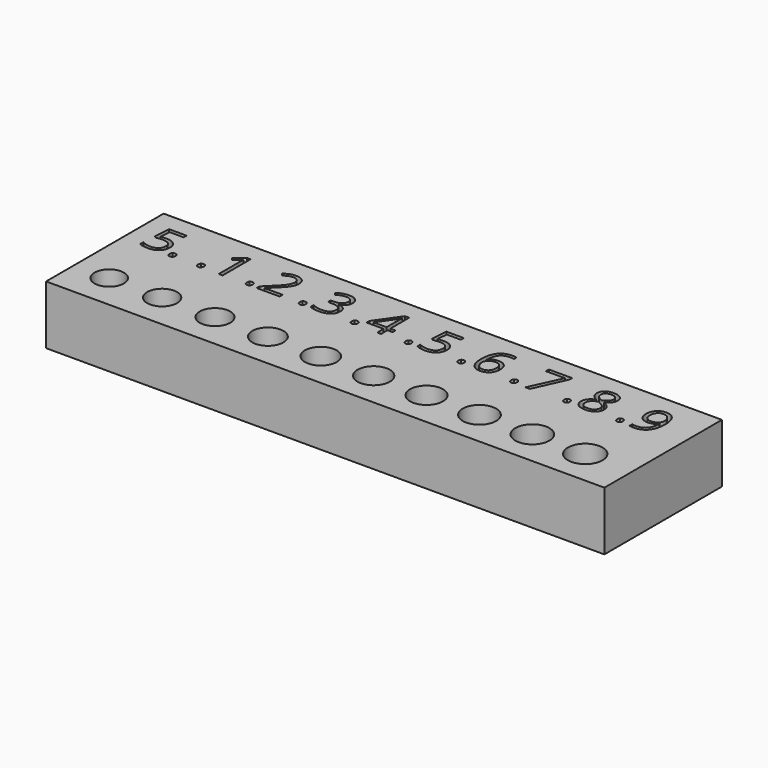
from build123d import *

# Parameters (mm, degrees)
F0_W         = 95
F0_H         = 25
F0_R         = 2.5
F0_R_2       = 2.55
F0_R_3       = 2.6
F0_R_4       = 2.65
F0_R_5       = 2.7
F0_R_6       = 2.75
F0_R_7       = 2.8
F0_R_8       = 2.85
F0_R_9       = 2.9
F0_R_10      = 2.95
F0_TEXT_SIZE = 8.3333333333
F1_DEPTH     = 8
F2_DEPTH     = 2
F3_DEPTH     = 4


# Not quite as in the source:
# - Text() gives the source's letters only with a copy of the font that has no kerning and outlines rounded to 1/6400 em; it was checked with that copy


with BuildPart() as f1:
    # F0 (on Top) → F1 (new body)
    with BuildSketch(Plane.XY):
        with Locations((47.5, 12.5)):
            Rectangle(F0_W, F0_H)
        with Locations((5.94223227, 6)):
            Circle(F0_R, mode=Mode.SUBTRACT)
        with Locations((14.94223227, 6)):
            Circle(F0_R_2, mode=Mode.SUBTRACT)
        with Locations((23.94223227, 6)):
            Circle(F0_R_3, mode=Mode.SUBTRACT)
        with Locations((32.94223227, 6)):
            Circle(F0_R_4, mode=Mode.SUBTRACT)
        with Locations((41.94223227, 6)):
            Circle(F0_R_5, mode=Mode.SUBTRACT)
        with Locations((50.94223227, 6)):
            Circle(F0_R_6, mode=Mode.SUBTRACT)
        with Locations((59.94223227, 6)):
            Circle(F0_R_7, mode=Mode.SUBTRACT)
        with Locations((68.94223227, 6)):
            Circle(F0_R_8, mode=Mode.SUBTRACT)
        with Locations((77.94223227, 6)):
            Circle(F0_R_9, mode=Mode.SUBTRACT)
        with Locations((86.94223227, 6)):
            Circle(F0_R_10, mode=Mode.SUBTRACT)
        with BuildLine():
            add(Edge.make_bspline(
                [(8.0092895616, 16.009765625), (7.8732218533, 16.1380208333), (7.8732218533, 16.4309895833)],
                knots=[0, 0, 0, 1, 1, 1], degree=2))
            add(Edge.make_bspline(
                [(7.8732218533, 16.4309895833), (7.8732218533, 16.7044270833), (7.9975708116, 16.8444010417)],
                knots=[0, 0, 0, 1, 1, 1], degree=2))
            add(Edge.make_bspline(
                [(7.9975708116, 16.8444010417), (8.12191977, 16.984375), (8.3536906033, 16.984375)],
                knots=[0, 0, 0, 1, 1, 1], degree=2))
            add(Edge.make_bspline(
                [(8.3536906033, 16.984375), (8.5893676866, 16.984375), (8.721529145, 16.8444010417)],
                knots=[0, 0, 0, 1, 1, 1], degree=2))
            add(Edge.make_bspline(
                [(8.721529145, 16.8444010417), (8.8536906033, 16.7044270833), (8.8536906033, 16.4309895833)],
                knots=[0, 0, 0, 1, 1, 1], degree=2))
            add(Edge.make_bspline(
                [(8.8536906033, 16.4309895833), (8.8536906033, 16.1666666667), (8.71957602, 16.0240885417)],
                knots=[0, 0, 0, 1, 1, 1], degree=2))
            add(Edge.make_bspline(
                [(8.71957602, 16.0240885417), (8.5854614366, 15.8815104167), (8.3536906033, 15.8815104167)],
                knots=[0, 0, 0, 1, 1, 1], degree=2))
            add(Edge.make_bspline(
                [(8.3536906033, 15.8815104167), (8.14535727, 15.8815104167), (8.0092895616, 16.009765625)],
                knots=[0, 0, 0, 1, 1, 1], degree=2))
        make_face(mode=Mode.SUBTRACT)
        with BuildLine():
            add(Edge.make_bspline(
                [(12.8634562283, 16.009765625), (12.72738852, 16.1380208333), (12.72738852, 16.4309895833)],
                knots=[0, 0, 0, 1, 1, 1], degree=2))
            add(Edge.make_bspline(
                [(12.72738852, 16.4309895833), (12.72738852, 16.7044270833), (12.8517374783, 16.8444010417)],
                knots=[0, 0, 0, 1, 1, 1], degree=2))
            add(Edge.make_bspline(
                [(12.8517374783, 16.8444010417), (12.9760864366, 16.984375), (13.20785727, 16.984375)],
                knots=[0, 0, 0, 1, 1, 1], degree=2))
            add(Edge.make_bspline(
                [(13.20785727, 16.984375), (13.4435343533, 16.984375), (13.5756958116, 16.8444010417)],
                knots=[0, 0, 0, 1, 1, 1], degree=2))
            add(Edge.make_bspline(
                [(13.5756958116, 16.8444010417), (13.70785727, 16.7044270833), (13.70785727, 16.4309895833)],
                knots=[0, 0, 0, 1, 1, 1], degree=2))
            add(Edge.make_bspline(
                [(13.70785727, 16.4309895833), (13.70785727, 16.1666666667), (13.5737426866, 16.0240885417)],
                knots=[0, 0, 0, 1, 1, 1], degree=2))
            add(Edge.make_bspline(
                [(13.5737426866, 16.0240885417), (13.4396281033, 15.8815104167), (13.20785727, 15.8815104167)],
                knots=[0, 0, 0, 1, 1, 1], degree=2))
            add(Edge.make_bspline(
                [(13.20785727, 15.8815104167), (12.9995239366, 15.8815104167), (12.8634562283, 16.009765625)],
                knots=[0, 0, 0, 1, 1, 1], degree=2))
        make_face(mode=Mode.SUBTRACT)
        with BuildLine():
            add(Edge.make_bspline(
                [(21.159029145, 16.009765625), (21.0229614366, 16.1380208333), (21.0229614366, 16.4309895833)],
                knots=[0, 0, 0, 1, 1, 1], degree=2))
            add(Edge.make_bspline(
                [(21.0229614366, 16.4309895833), (21.0229614366, 16.7044270833), (21.147310395, 16.8444010417)],
                knots=[0, 0, 0, 1, 1, 1], degree=2))
            add(Edge.make_bspline(
                [(21.147310395, 16.8444010417), (21.2716593533, 16.984375), (21.5034301866, 16.984375)],
                knots=[0, 0, 0, 1, 1, 1], degree=2))
            add(Edge.make_bspline(
                [(21.5034301866, 16.984375), (21.73910727, 16.984375), (21.8712687283, 16.8444010417)],
                knots=[0, 0, 0, 1, 1, 1], degree=2))
            add(Edge.make_bspline(
                [(21.8712687283, 16.8444010417), (22.0034301866, 16.7044270833), (22.0034301866, 16.4309895833)],
                knots=[0, 0, 0, 1, 1, 1], degree=2))
            add(Edge.make_bspline(
                [(22.0034301866, 16.4309895833), (22.0034301866, 16.1666666667), (21.8693156033, 16.0240885417)],
                knots=[0, 0, 0, 1, 1, 1], degree=2))
            add(Edge.make_bspline(
                [(21.8693156033, 16.0240885417), (21.73520102, 15.8815104167), (21.5034301866, 15.8815104167)],
                knots=[0, 0, 0, 1, 1, 1], degree=2))
            add(Edge.make_bspline(
                [(21.5034301866, 15.8815104167), (21.2950968533, 15.8815104167), (21.159029145, 16.009765625)],
                knots=[0, 0, 0, 1, 1, 1], degree=2))
        make_face(mode=Mode.SUBTRACT)
        with BuildLine():
            add(Edge.make_bspline(
                [(30.1798624783, 16.009765625), (30.04379477, 16.1380208333), (30.04379477, 16.4309895833)],
                knots=[0, 0, 0, 1, 1, 1], degree=2))
            add(Edge.make_bspline(
                [(30.04379477, 16.4309895833), (30.04379477, 16.7044270833), (30.1681437283, 16.8444010417)],
                knots=[0, 0, 0, 1, 1, 1], degree=2))
            add(Edge.make_bspline(
                [(30.1681437283, 16.8444010417), (30.2924926866, 16.984375), (30.52426352, 16.984375)],
                knots=[0, 0, 0, 1, 1, 1], degree=2))
            add(Edge.make_bspline(
                [(30.52426352, 16.984375), (30.7599406033, 16.984375), (30.8921020616, 16.8444010417)],
                knots=[0, 0, 0, 1, 1, 1], degree=2))
            add(Edge.make_bspline(
                [(30.8921020616, 16.8444010417), (31.02426352, 16.7044270833), (31.02426352, 16.4309895833)],
                knots=[0, 0, 0, 1, 1, 1], degree=2))
            add(Edge.make_bspline(
                [(31.02426352, 16.4309895833), (31.02426352, 16.1666666667), (30.8901489366, 16.0240885417)],
                knots=[0, 0, 0, 1, 1, 1], degree=2))
            add(Edge.make_bspline(
                [(30.8901489366, 16.0240885417), (30.7560343533, 15.8815104167), (30.52426352, 15.8815104167)],
                knots=[0, 0, 0, 1, 1, 1], degree=2))
            add(Edge.make_bspline(
                [(30.52426352, 15.8815104167), (30.3159301866, 15.8815104167), (30.1798624783, 16.009765625)],
                knots=[0, 0, 0, 1, 1, 1], degree=2))
        make_face(mode=Mode.SUBTRACT)
        with BuildLine():
            add(Edge.make_bspline(
                [(39.0190551866, 16.009765625), (38.8829874783, 16.1380208333), (38.8829874783, 16.4309895833)],
                knots=[0, 0, 0, 1, 1, 1], degree=2))
            add(Edge.make_bspline(
                [(38.8829874783, 16.4309895833), (38.8829874783, 16.7044270833), (39.0073364366, 16.8444010417)],
                knots=[0, 0, 0, 1, 1, 1], degree=2))
            add(Edge.make_bspline(
                [(39.0073364366, 16.8444010417), (39.131685395, 16.984375), (39.3634562283, 16.984375)],
                knots=[0, 0, 0, 1, 1, 1], degree=2))
            add(Edge.make_bspline(
                [(39.3634562283, 16.984375), (39.5991333116, 16.984375), (39.73129477, 16.8444010417)],
                knots=[0, 0, 0, 1, 1, 1], degree=2))
            add(Edge.make_bspline(
                [(39.73129477, 16.8444010417), (39.8634562283, 16.7044270833), (39.8634562283, 16.4309895833)],
                knots=[0, 0, 0, 1, 1, 1], degree=2))
            add(Edge.make_bspline(
                [(39.8634562283, 16.4309895833), (39.8634562283, 16.1666666667), (39.729341645, 16.0240885417)],
                knots=[0, 0, 0, 1, 1, 1], degree=2))
            add(Edge.make_bspline(
                [(39.729341645, 16.0240885417), (39.5952270616, 15.8815104167), (39.3634562283, 15.8815104167)],
                knots=[0, 0, 0, 1, 1, 1], degree=2))
            add(Edge.make_bspline(
                [(39.3634562283, 15.8815104167), (39.155122895, 15.8815104167), (39.0190551866, 16.009765625)],
                knots=[0, 0, 0, 1, 1, 1], degree=2))
        make_face(mode=Mode.SUBTRACT)
        with BuildLine():
            add(Edge.make_bspline(
                [(3.82504477, 19.5403645833), (4.2924926866, 19.6341145833), (4.7573364366, 19.6341145833)],
                knots=[0, 0, 0, 1, 1, 1], degree=2))
            add(Edge.make_bspline(
                [(4.7573364366, 19.6341145833), (5.6974406033, 19.6341145833), (6.2365031033, 19.16796875)],
                knots=[0, 0, 0, 1, 1, 1], degree=2))
            add(Edge.make_bspline(
                [(6.2365031033, 19.16796875), (6.7755656033, 18.7018229167), (6.7755656033, 17.8919270833)],
                knots=[0, 0, 0, 1, 1, 1], degree=2))
            add(Edge.make_bspline(
                [(6.7755656033, 17.8919270833), (6.7755656033, 16.96875), (6.1876749783, 16.443359375)],
                knots=[0, 0, 0, 1, 1, 1], degree=2))
            add(Edge.make_bspline(
                [(6.1876749783, 16.443359375), (5.5997843533, 15.91796875), (4.5659301866, 15.91796875)],
                knots=[0, 0, 0, 1, 1, 1], degree=2))
            add(Edge.make_bspline(
                [(4.5659301866, 15.91796875), (3.5607218533, 15.91796875), (3.03207602, 16.2395833333)],
                knots=[0, 0, 0, 1, 1, 1], degree=2))
            Line((3.03207602, 16.2395833333), (3.03207602, 16.890625))
            add(Edge.make_bspline(
                [(3.03207602, 16.890625), (3.3159301866, 16.7083333333), (3.73910727, 16.6041666667)],
                knots=[0, 0, 0, 1, 1, 1], degree=2))
            add(Edge.make_bspline(
                [(3.73910727, 16.6041666667), (4.1622843533, 16.5), (4.5737426866, 16.5)],
                knots=[0, 0, 0, 1, 1, 1], degree=2))
            add(Edge.make_bspline(
                [(4.5737426866, 16.5), (5.28988852, 16.5), (5.686372895, 16.837890625)],
                knots=[0, 0, 0, 1, 1, 1], degree=2))
            add(Edge.make_bspline(
                [(5.686372895, 16.837890625), (6.08285727, 17.17578125), (6.08285727, 17.8151041667)],
                knots=[0, 0, 0, 1, 1, 1], degree=2))
            add(Edge.make_bspline(
                [(6.08285727, 17.8151041667), (6.08285727, 19.0598958333), (4.5581176866, 19.0598958333)],
                knots=[0, 0, 0, 1, 1, 1], degree=2))
            add(Edge.make_bspline(
                [(4.5581176866, 19.0598958333), (4.1713989366, 19.0598958333), (3.52426352, 18.94140625)],
                knots=[0, 0, 0, 1, 1, 1], degree=2))
            Line((3.52426352, 18.94140625), (3.1740031033, 19.1653645833))
            Line((3.1740031033, 19.1653645833), (3.3979614366, 21.94921875))
            Line((3.3979614366, 21.94921875), (6.35629477, 21.94921875))
            Line((6.35629477, 21.94921875), (6.35629477, 21.3268229167))
            Line((6.35629477, 21.3268229167), (3.9760864366, 21.3268229167))
            Line((3.9760864366, 21.3268229167), (3.82504477, 19.5403645833))
        make_face(mode=Mode.SUBTRACT)
        with BuildLine():
            Line((17.23520102, 21.94921875), (17.23520102, 16))
            Line((17.23520102, 16), (16.5763468533, 16))
            Line((16.5763468533, 16), (16.5763468533, 20.2395833333))
            add(Edge.make_bspline(
                [(16.5763468533, 20.2395833333), (16.5763468533, 20.76953125), (16.6088989366, 21.2408854167)],
                knots=[0, 0, 0, 1, 1, 1], degree=2))
            add(Edge.make_bspline(
                [(16.6088989366, 21.2408854167), (16.52426352, 21.1549479167), (16.4181437283, 21.0618489583)],
                knots=[0, 0, 0, 1, 1, 1], degree=2))
            add(Edge.make_bspline(
                [(16.4181437283, 21.0618489583), (16.3120239366, 20.96875), (15.45004477, 20.2682291667)],
                knots=[0, 0, 0, 1, 1, 1], degree=2))
            Line((15.45004477, 20.2682291667), (15.0919718533, 20.7317708333))
            Line((15.0919718533, 20.7317708333), (16.6661906033, 21.94921875))
            Line((16.6661906033, 21.94921875), (17.23520102, 21.94921875))
        make_face(mode=Mode.SUBTRACT)
        with BuildLine():
            Line((26.9396281033, 16.6263020833), (26.9396281033, 16))
            Line((26.9396281033, 16), (23.0294718533, 16))
            Line((23.0294718533, 16), (23.0294718533, 16.58203125))
            Line((23.0294718533, 16.58203125), (24.5958781033, 18.15625))
            add(Edge.make_bspline(
                [(24.5958781033, 18.15625), (25.3120239366, 18.8815104167), (25.53988852, 19.1907552083)],
                knots=[0, 0, 0, 1, 1, 1], degree=2))
            add(Edge.make_bspline(
                [(25.53988852, 19.1907552083), (25.7677531033, 19.5), (25.881685395, 19.79296875)],
                knots=[0, 0, 0, 1, 1, 1], degree=2))
            add(Edge.make_bspline(
                [(25.881685395, 19.79296875), (25.9956176866, 20.0859375), (25.9956176866, 20.4231770833)],
                knots=[0, 0, 0, 1, 1, 1], degree=2))
            add(Edge.make_bspline(
                [(25.9956176866, 20.4231770833), (25.9956176866, 20.8997395833), (25.7065551866, 21.1783854167)],
                knots=[0, 0, 0, 1, 1, 1], degree=2))
            add(Edge.make_bspline(
                [(25.7065551866, 21.1783854167), (25.4174926866, 21.45703125), (24.9044718533, 21.45703125)],
                knots=[0, 0, 0, 1, 1, 1], degree=2))
            add(Edge.make_bspline(
                [(24.9044718533, 21.45703125), (24.5346801866, 21.45703125), (24.2026489366, 21.3346354167)],
                knots=[0, 0, 0, 1, 1, 1], degree=2))
            add(Edge.make_bspline(
                [(24.2026489366, 21.3346354167), (23.8706176866, 21.2122395833), (23.4643676866, 20.890625)],
                knots=[0, 0, 0, 1, 1, 1], degree=2))
            Line((23.4643676866, 20.890625), (23.10629477, 21.3502604167))
            add(Edge.make_bspline(
                [(23.10629477, 21.3502604167), (23.9279093533, 22.0338541667), (24.8966593533, 22.0338541667)],
                knots=[0, 0, 0, 1, 1, 1], degree=2))
            add(Edge.make_bspline(
                [(24.8966593533, 22.0338541667), (25.73520102, 22.0338541667), (26.2111124783, 21.6048177083)],
                knots=[0, 0, 0, 1, 1, 1], degree=2))
            add(Edge.make_bspline(
                [(26.2111124783, 21.6048177083), (26.6870239366, 21.17578125), (26.6870239366, 20.4518229167)],
                knots=[0, 0, 0, 1, 1, 1], degree=2))
            add(Edge.make_bspline(
                [(26.6870239366, 20.4518229167), (26.6870239366, 19.8854166667), (26.3693156033, 19.33203125)],
                knots=[0, 0, 0, 1, 1, 1], degree=2))
            add(Edge.make_bspline(
                [(26.3693156033, 19.33203125), (26.05160727, 18.7786458333), (25.1818156033, 17.9322916667)],
                knots=[0, 0, 0, 1, 1, 1], degree=2))
            Line((25.1818156033, 17.9322916667), (23.87973227, 16.6588541667))
            Line((23.87973227, 16.6588541667), (23.87973227, 16.6263020833))
            Line((23.87973227, 16.6263020833), (26.9396281033, 16.6263020833))
        make_face(mode=Mode.SUBTRACT)
        with BuildLine():
            add(Edge.make_bspline(
                [(35.2560343533, 21.6373697917), (35.7365031033, 21.2408854167), (35.7365031033, 20.5494791667)],
                knots=[0, 0, 0, 1, 1, 1], degree=2))
            add(Edge.make_bspline(
                [(35.7365031033, 20.5494791667), (35.7365031033, 19.9791666667), (35.416841645, 19.6171875)],
                knots=[0, 0, 0, 1, 1, 1], degree=2))
            add(Edge.make_bspline(
                [(35.416841645, 19.6171875), (35.0971801866, 19.2552083333), (34.5112426866, 19.1328125)],
                knots=[0, 0, 0, 1, 1, 1], degree=2))
            Line((34.5112426866, 19.1328125), (34.5112426866, 19.1002604167))
            add(Edge.make_bspline(
                [(34.5112426866, 19.1002604167), (35.22738852, 19.01171875), (35.573091645, 18.6451822917)],
                knots=[0, 0, 0, 1, 1, 1], degree=2))
            add(Edge.make_bspline(
                [(35.573091645, 18.6451822917), (35.91879477, 18.2786458333), (35.91879477, 17.6848958333)],
                knots=[0, 0, 0, 1, 1, 1], degree=2))
            add(Edge.make_bspline(
                [(35.91879477, 17.6848958333), (35.91879477, 16.8346354167), (35.32895102, 16.3763020833)],
                knots=[0, 0, 0, 1, 1, 1], degree=2))
            add(Edge.make_bspline(
                [(35.32895102, 16.3763020833), (34.73910727, 15.91796875), (33.65316977, 15.91796875)],
                knots=[0, 0, 0, 1, 1, 1], degree=2))
            add(Edge.make_bspline(
                [(33.65316977, 15.91796875), (33.18051352, 15.91796875), (32.787935395, 15.9895833333)],
                knots=[0, 0, 0, 1, 1, 1], degree=2))
            add(Edge.make_bspline(
                [(32.787935395, 15.9895833333), (32.39535727, 16.0611979167), (32.0255656033, 16.2395833333)],
                knots=[0, 0, 0, 1, 1, 1], degree=2))
            Line((32.0255656033, 16.2395833333), (32.0255656033, 16.8828125))
            add(Edge.make_bspline(
                [(32.0255656033, 16.8828125), (32.4122843533, 16.69140625), (32.8497843533, 16.591796875)],
                knots=[0, 0, 0, 1, 1, 1], degree=2))
            add(Edge.make_bspline(
                [(32.8497843533, 16.591796875), (33.2872843533, 16.4921875), (33.6779093533, 16.4921875)],
                knots=[0, 0, 0, 1, 1, 1], degree=2))
            add(Edge.make_bspline(
                [(33.6779093533, 16.4921875), (35.21957602, 16.4921875), (35.21957602, 17.7005208333)],
                knots=[0, 0, 0, 1, 1, 1], degree=2))
            add(Edge.make_bspline(
                [(35.21957602, 17.7005208333), (35.21957602, 18.7838541667), (33.5190551866, 18.7838541667)],
                knots=[0, 0, 0, 1, 1, 1], degree=2))
            Line((33.5190551866, 18.7838541667), (32.9331176866, 18.7838541667))
            Line((32.9331176866, 18.7838541667), (32.9331176866, 19.3645833333))
            Line((32.9331176866, 19.3645833333), (33.5268676866, 19.3645833333))
            add(Edge.make_bspline(
                [(33.5268676866, 19.3645833333), (34.2221801866, 19.3645833333), (34.6290812283, 19.671875)],
                knots=[0, 0, 0, 1, 1, 1], degree=2))
            add(Edge.make_bspline(
                [(34.6290812283, 19.671875), (35.03598227, 19.9791666667), (35.03598227, 20.5247395833)],
                knots=[0, 0, 0, 1, 1, 1], degree=2))
            add(Edge.make_bspline(
                [(35.03598227, 20.5247395833), (35.03598227, 20.9596354167), (34.737154145, 21.2083333333)],
                knots=[0, 0, 0, 1, 1, 1], degree=2))
            add(Edge.make_bspline(
                [(34.737154145, 21.2083333333), (34.43832602, 21.45703125), (33.9253051866, 21.45703125)],
                knots=[0, 0, 0, 1, 1, 1], degree=2))
            add(Edge.make_bspline(
                [(33.9253051866, 21.45703125), (33.5346801866, 21.45703125), (33.1889770616, 21.3509114583)],
                knots=[0, 0, 0, 1, 1, 1], degree=2))
            add(Edge.make_bspline(
                [(33.1889770616, 21.3509114583), (32.8432739366, 21.2447916667), (32.39926352, 20.9596354167)],
                knots=[0, 0, 0, 1, 1, 1], degree=2))
            Line((32.39926352, 20.9596354167), (32.0581176866, 21.4153645833))
            add(Edge.make_bspline(
                [(32.0581176866, 21.4153645833), (32.4240031033, 21.7044270833), (32.9018676866, 21.869140625)],
                knots=[0, 0, 0, 1, 1, 1], degree=2))
            add(Edge.make_bspline(
                [(32.9018676866, 21.869140625), (33.37973227, 22.0338541667), (33.9096801866, 22.0338541667)],
                knots=[0, 0, 0, 1, 1, 1], degree=2))
            add(Edge.make_bspline(
                [(33.9096801866, 22.0338541667), (34.7755656033, 22.0338541667), (35.2560343533, 21.6373697917)],
                knots=[0, 0, 0, 1, 1, 1], degree=2))
        make_face(mode=Mode.SUBTRACT)
        Polygon((45.0796020616, 17.9817708333), (45.0796020616, 17.3671875), (44.1967895616, 17.3671875), (44.1967895616, 16), (43.549654145, 16), (43.549654145, 17.3671875), (40.6564249783, 17.3671875), (40.6564249783, 17.95703125), (43.4806437283, 21.9817708333), (44.1967895616, 21.9817708333), (44.1967895616, 17.9817708333), align=None, mode=Mode.SUBTRACT)
        with BuildLine():
            add(Edge.make_bspline(
                [(48.1753051866, 16.009765625), (48.0392374783, 16.1380208333), (48.0392374783, 16.4309895833)],
                knots=[0, 0, 0, 1, 1, 1], degree=2))
            add(Edge.make_bspline(
                [(48.0392374783, 16.4309895833), (48.0392374783, 16.7044270833), (48.1635864366, 16.8444010417)],
                knots=[0, 0, 0, 1, 1, 1], degree=2))
            add(Edge.make_bspline(
                [(48.1635864366, 16.8444010417), (48.287935395, 16.984375), (48.5197062283, 16.984375)],
                knots=[0, 0, 0, 1, 1, 1], degree=2))
            add(Edge.make_bspline(
                [(48.5197062283, 16.984375), (48.7553833116, 16.984375), (48.88754477, 16.8444010417)],
                knots=[0, 0, 0, 1, 1, 1], degree=2))
            add(Edge.make_bspline(
                [(48.88754477, 16.8444010417), (49.0197062283, 16.7044270833), (49.0197062283, 16.4309895833)],
                knots=[0, 0, 0, 1, 1, 1], degree=2))
            add(Edge.make_bspline(
                [(49.0197062283, 16.4309895833), (49.0197062283, 16.1666666667), (48.885591645, 16.0240885417)],
                knots=[0, 0, 0, 1, 1, 1], degree=2))
            add(Edge.make_bspline(
                [(48.885591645, 16.0240885417), (48.7514770616, 15.8815104167), (48.5197062283, 15.8815104167)],
                knots=[0, 0, 0, 1, 1, 1], degree=2))
            add(Edge.make_bspline(
                [(48.5197062283, 15.8815104167), (48.311372895, 15.8815104167), (48.1753051866, 16.009765625)],
                knots=[0, 0, 0, 1, 1, 1], degree=2))
        make_face(mode=Mode.SUBTRACT)
        with BuildLine():
            add(Edge.make_bspline(
                [(57.1388468533, 16.009765625), (57.002779145, 16.1380208333), (57.002779145, 16.4309895833)],
                knots=[0, 0, 0, 1, 1, 1], degree=2))
            add(Edge.make_bspline(
                [(57.002779145, 16.4309895833), (57.002779145, 16.7044270833), (57.1271281033, 16.8444010417)],
                knots=[0, 0, 0, 1, 1, 1], degree=2))
            add(Edge.make_bspline(
                [(57.1271281033, 16.8444010417), (57.2514770616, 16.984375), (57.483247895, 16.984375)],
                knots=[0, 0, 0, 1, 1, 1], degree=2))
            add(Edge.make_bspline(
                [(57.483247895, 16.984375), (57.7189249783, 16.984375), (57.8510864366, 16.8444010417)],
                knots=[0, 0, 0, 1, 1, 1], degree=2))
            add(Edge.make_bspline(
                [(57.8510864366, 16.8444010417), (57.983247895, 16.7044270833), (57.983247895, 16.4309895833)],
                knots=[0, 0, 0, 1, 1, 1], degree=2))
            add(Edge.make_bspline(
                [(57.983247895, 16.4309895833), (57.983247895, 16.1666666667), (57.8491333116, 16.0240885417)],
                knots=[0, 0, 0, 1, 1, 1], degree=2))
            add(Edge.make_bspline(
                [(57.8491333116, 16.0240885417), (57.7150187283, 15.8815104167), (57.483247895, 15.8815104167)],
                knots=[0, 0, 0, 1, 1, 1], degree=2))
            add(Edge.make_bspline(
                [(57.483247895, 15.8815104167), (57.2749145616, 15.8815104167), (57.1388468533, 16.009765625)],
                knots=[0, 0, 0, 1, 1, 1], degree=2))
        make_face(mode=Mode.SUBTRACT)
        with BuildLine():
            add(Edge.make_bspline(
                [(66.147310395, 16.009765625), (66.0112426866, 16.1380208333), (66.0112426866, 16.4309895833)],
                knots=[0, 0, 0, 1, 1, 1], degree=2))
            add(Edge.make_bspline(
                [(66.0112426866, 16.4309895833), (66.0112426866, 16.7044270833), (66.135591645, 16.8444010417)],
                knots=[0, 0, 0, 1, 1, 1], degree=2))
            add(Edge.make_bspline(
                [(66.135591645, 16.8444010417), (66.2599406033, 16.984375), (66.4917114366, 16.984375)],
                knots=[0, 0, 0, 1, 1, 1], degree=2))
            add(Edge.make_bspline(
                [(66.4917114366, 16.984375), (66.72738852, 16.984375), (66.8595499783, 16.8444010417)],
                knots=[0, 0, 0, 1, 1, 1], degree=2))
            add(Edge.make_bspline(
                [(66.8595499783, 16.8444010417), (66.9917114366, 16.7044270833), (66.9917114366, 16.4309895833)],
                knots=[0, 0, 0, 1, 1, 1], degree=2))
            add(Edge.make_bspline(
                [(66.9917114366, 16.4309895833), (66.9917114366, 16.1666666667), (66.8575968533, 16.0240885417)],
                knots=[0, 0, 0, 1, 1, 1], degree=2))
            add(Edge.make_bspline(
                [(66.8575968533, 16.0240885417), (66.72348227, 15.8815104167), (66.4917114366, 15.8815104167)],
                knots=[0, 0, 0, 1, 1, 1], degree=2))
            add(Edge.make_bspline(
                [(66.4917114366, 15.8815104167), (66.2833781033, 15.8815104167), (66.147310395, 16.009765625)],
                knots=[0, 0, 0, 1, 1, 1], degree=2))
        make_face(mode=Mode.SUBTRACT)
        with BuildLine():
            add(Edge.make_bspline(
                [(75.151216645, 16.009765625), (75.0151489366, 16.1380208333), (75.0151489366, 16.4309895833)],
                knots=[0, 0, 0, 1, 1, 1], degree=2))
            add(Edge.make_bspline(
                [(75.0151489366, 16.4309895833), (75.0151489366, 16.7044270833), (75.139497895, 16.8444010417)],
                knots=[0, 0, 0, 1, 1, 1], degree=2))
            add(Edge.make_bspline(
                [(75.139497895, 16.8444010417), (75.2638468533, 16.984375), (75.4956176866, 16.984375)],
                knots=[0, 0, 0, 1, 1, 1], degree=2))
            add(Edge.make_bspline(
                [(75.4956176866, 16.984375), (75.73129477, 16.984375), (75.8634562283, 16.8444010417)],
                knots=[0, 0, 0, 1, 1, 1], degree=2))
            add(Edge.make_bspline(
                [(75.8634562283, 16.8444010417), (75.9956176866, 16.7044270833), (75.9956176866, 16.4309895833)],
                knots=[0, 0, 0, 1, 1, 1], degree=2))
            add(Edge.make_bspline(
                [(75.9956176866, 16.4309895833), (75.9956176866, 16.1666666667), (75.8615031033, 16.0240885417)],
                knots=[0, 0, 0, 1, 1, 1], degree=2))
            add(Edge.make_bspline(
                [(75.8615031033, 16.0240885417), (75.72738852, 15.8815104167), (75.4956176866, 15.8815104167)],
                knots=[0, 0, 0, 1, 1, 1], degree=2))
            add(Edge.make_bspline(
                [(75.4956176866, 15.8815104167), (75.2872843533, 15.8815104167), (75.151216645, 16.009765625)],
                knots=[0, 0, 0, 1, 1, 1], degree=2))
        make_face(mode=Mode.SUBTRACT)
        with BuildLine():
            add(Edge.make_bspline(
                [(84.159029145, 16.009765625), (84.0229614366, 16.1380208333), (84.0229614366, 16.4309895833)],
                knots=[0, 0, 0, 1, 1, 1], degree=2))
            add(Edge.make_bspline(
                [(84.0229614366, 16.4309895833), (84.0229614366, 16.7044270833), (84.147310395, 16.8444010417)],
                knots=[0, 0, 0, 1, 1, 1], degree=2))
            add(Edge.make_bspline(
                [(84.147310395, 16.8444010417), (84.2716593533, 16.984375), (84.5034301866, 16.984375)],
                knots=[0, 0, 0, 1, 1, 1], degree=2))
            add(Edge.make_bspline(
                [(84.5034301866, 16.984375), (84.73910727, 16.984375), (84.8712687283, 16.8444010417)],
                knots=[0, 0, 0, 1, 1, 1], degree=2))
            add(Edge.make_bspline(
                [(84.8712687283, 16.8444010417), (85.0034301866, 16.7044270833), (85.0034301866, 16.4309895833)],
                knots=[0, 0, 0, 1, 1, 1], degree=2))
            add(Edge.make_bspline(
                [(85.0034301866, 16.4309895833), (85.0034301866, 16.1666666667), (84.8693156033, 16.0240885417)],
                knots=[0, 0, 0, 1, 1, 1], degree=2))
            add(Edge.make_bspline(
                [(84.8693156033, 16.0240885417), (84.73520102, 15.8815104167), (84.5034301866, 15.8815104167)],
                knots=[0, 0, 0, 1, 1, 1], degree=2))
            add(Edge.make_bspline(
                [(84.5034301866, 15.8815104167), (84.2950968533, 15.8815104167), (84.159029145, 16.009765625)],
                knots=[0, 0, 0, 1, 1, 1], degree=2))
        make_face(mode=Mode.SUBTRACT)
        with BuildLine():
            add(Edge.make_bspline(
                [(50.9728312283, 19.5403645833), (51.440279145, 19.6341145833), (51.905122895, 19.6341145833)],
                knots=[0, 0, 0, 1, 1, 1], degree=2))
            add(Edge.make_bspline(
                [(51.905122895, 19.6341145833), (52.8452270616, 19.6341145833), (53.3842895616, 19.16796875)],
                knots=[0, 0, 0, 1, 1, 1], degree=2))
            add(Edge.make_bspline(
                [(53.3842895616, 19.16796875), (53.9233520616, 18.7018229167), (53.9233520616, 17.8919270833)],
                knots=[0, 0, 0, 1, 1, 1], degree=2))
            add(Edge.make_bspline(
                [(53.9233520616, 17.8919270833), (53.9233520616, 16.96875), (53.3354614366, 16.443359375)],
                knots=[0, 0, 0, 1, 1, 1], degree=2))
            add(Edge.make_bspline(
                [(53.3354614366, 16.443359375), (52.7475708116, 15.91796875), (51.713716645, 15.91796875)],
                knots=[0, 0, 0, 1, 1, 1], degree=2))
            add(Edge.make_bspline(
                [(51.713716645, 15.91796875), (50.7085083116, 15.91796875), (50.1798624783, 16.2395833333)],
                knots=[0, 0, 0, 1, 1, 1], degree=2))
            Line((50.1798624783, 16.2395833333), (50.1798624783, 16.890625))
            add(Edge.make_bspline(
                [(50.1798624783, 16.890625), (50.463716645, 16.7083333333), (50.8868937283, 16.6041666667)],
                knots=[0, 0, 0, 1, 1, 1], degree=2))
            add(Edge.make_bspline(
                [(50.8868937283, 16.6041666667), (51.3100708116, 16.5), (51.721529145, 16.5)],
                knots=[0, 0, 0, 1, 1, 1], degree=2))
            add(Edge.make_bspline(
                [(51.721529145, 16.5), (52.4376749783, 16.5), (52.8341593533, 16.837890625)],
                knots=[0, 0, 0, 1, 1, 1], degree=2))
            add(Edge.make_bspline(
                [(52.8341593533, 16.837890625), (53.2306437283, 17.17578125), (53.2306437283, 17.8151041667)],
                knots=[0, 0, 0, 1, 1, 1], degree=2))
            add(Edge.make_bspline(
                [(53.2306437283, 17.8151041667), (53.2306437283, 19.0598958333), (51.705904145, 19.0598958333)],
                knots=[0, 0, 0, 1, 1, 1], degree=2))
            add(Edge.make_bspline(
                [(51.705904145, 19.0598958333), (51.319185395, 19.0598958333), (50.6720499783, 18.94140625)],
                knots=[0, 0, 0, 1, 1, 1], degree=2))
            Line((50.6720499783, 18.94140625), (50.3217895616, 19.1653645833))
            Line((50.3217895616, 19.1653645833), (50.545747895, 21.94921875))
            Line((50.545747895, 21.94921875), (53.5040812283, 21.94921875))
            Line((53.5040812283, 21.94921875), (53.5040812283, 21.3268229167))
            Line((53.5040812283, 21.3268229167), (51.123872895, 21.3268229167))
            Line((51.123872895, 21.3268229167), (50.9728312283, 19.5403645833))
        make_face(mode=Mode.SUBTRACT)
        with BuildLine():
            add(Edge.make_bspline(
                [(59.6193156033, 16.6119791667), (59.0782999783, 17.3059895833), (59.0782999783, 18.54296875)],
                knots=[0, 0, 0, 1, 1, 1], degree=2))
            add(Edge.make_bspline(
                [(59.0782999783, 18.54296875), (59.0782999783, 20.296875), (59.7599406033, 21.1653645833)],
                knots=[0, 0, 0, 1, 1, 1], degree=2))
            add(Edge.make_bspline(
                [(59.7599406033, 21.1653645833), (60.4415812283, 22.0338541667), (61.776216645, 22.0338541667)],
                knots=[0, 0, 0, 1, 1, 1], degree=2))
            add(Edge.make_bspline(
                [(61.776216645, 22.0338541667), (62.2358520616, 22.0338541667), (62.5001749783, 21.95703125)],
                knots=[0, 0, 0, 1, 1, 1], degree=2))
            Line((62.5001749783, 21.95703125), (62.5001749783, 21.375))
            add(Edge.make_bspline(
                [(62.5001749783, 21.375), (62.186372895, 21.4765625), (61.784029145, 21.4765625)],
                knots=[0, 0, 0, 1, 1, 1], degree=2))
            add(Edge.make_bspline(
                [(61.784029145, 21.4765625), (60.826997895, 21.4765625), (60.3224406033, 20.880859375)],
                knots=[0, 0, 0, 1, 1, 1], degree=2))
            add(Edge.make_bspline(
                [(60.3224406033, 20.880859375), (59.8178833116, 20.28515625), (59.7697062283, 19.0065104167)],
                knots=[0, 0, 0, 1, 1, 1], degree=2))
            Line((59.7697062283, 19.0065104167), (59.8178833116, 19.0065104167))
            add(Edge.make_bspline(
                [(59.8178833116, 19.0065104167), (60.2657999783, 19.70703125), (61.2345499783, 19.70703125)],
                knots=[0, 0, 0, 1, 1, 1], degree=2))
            add(Edge.make_bspline(
                [(61.2345499783, 19.70703125), (62.0366333116, 19.70703125), (62.4982218533, 19.22265625)],
                knots=[0, 0, 0, 1, 1, 1], degree=2))
            add(Edge.make_bspline(
                [(62.4982218533, 19.22265625), (62.959810395, 18.73828125), (62.959810395, 17.9088541667)],
                knots=[0, 0, 0, 1, 1, 1], degree=2))
            add(Edge.make_bspline(
                [(62.959810395, 17.9088541667), (62.959810395, 16.98046875), (62.4532999783, 16.44921875)],
                knots=[0, 0, 0, 1, 1, 1], degree=2))
            add(Edge.make_bspline(
                [(62.4532999783, 16.44921875), (61.9467895616, 15.91796875), (61.0835083116, 15.91796875)],
                knots=[0, 0, 0, 1, 1, 1], degree=2))
            add(Edge.make_bspline(
                [(61.0835083116, 15.91796875), (60.1603312283, 15.91796875), (59.6193156033, 16.6119791667)],
                knots=[0, 0, 0, 1, 1, 1], degree=2))
        make_face(mode=Mode.SUBTRACT)
        Polygon((69.5190551866, 16), (68.77035727, 16), (71.23520102, 21.3268229167), (67.99301352, 21.3268229167), (67.99301352, 21.94921875), (71.9513468533, 21.94921875), (71.9513468533, 21.4075520833), align=None, mode=Mode.SUBTRACT)
        with BuildLine():
            add(Edge.make_bspline(
                [(77.7104614366, 21.6497395833), (78.18832602, 22.0338541667), (78.9904093533, 22.0338541667)],
                knots=[0, 0, 0, 1, 1, 1], degree=2))
            add(Edge.make_bspline(
                [(78.9904093533, 22.0338541667), (79.8042114366, 22.0338541667), (80.280122895, 21.6555989583)],
                knots=[0, 0, 0, 1, 1, 1], degree=2))
            add(Edge.make_bspline(
                [(80.280122895, 21.6555989583), (80.7560343533, 21.27734375), (80.7560343533, 20.6106770833)],
                knots=[0, 0, 0, 1, 1, 1], degree=2))
            add(Edge.make_bspline(
                [(80.7560343533, 20.6106770833), (80.7560343533, 20.1705729167), (80.4838989366, 19.80859375)],
                knots=[0, 0, 0, 1, 1, 1], degree=2))
            add(Edge.make_bspline(
                [(80.4838989366, 19.80859375), (80.21176352, 19.4466145833), (79.6128051866, 19.1497395833)],
                knots=[0, 0, 0, 1, 1, 1], degree=2))
            add(Edge.make_bspline(
                [(79.6128051866, 19.1497395833), (80.33676352, 18.8033854167), (80.6421020616, 18.4231770833)],
                knots=[0, 0, 0, 1, 1, 1], degree=2))
            add(Edge.make_bspline(
                [(80.6421020616, 18.4231770833), (80.9474406033, 18.04296875), (80.9474406033, 17.5416666667)],
                knots=[0, 0, 0, 1, 1, 1], degree=2))
            add(Edge.make_bspline(
                [(80.9474406033, 17.5416666667), (80.9474406033, 16.8020833333), (80.43051352, 16.3600260417)],
                knots=[0, 0, 0, 1, 1, 1], degree=2))
            add(Edge.make_bspline(
                [(80.43051352, 16.3600260417), (79.9135864366, 15.91796875), (79.0151489366, 15.91796875)],
                knots=[0, 0, 0, 1, 1, 1], degree=2))
            add(Edge.make_bspline(
                [(79.0151489366, 15.91796875), (78.06332602, 15.91796875), (77.5503051866, 16.3352864583)],
                knots=[0, 0, 0, 1, 1, 1], degree=2))
            add(Edge.make_bspline(
                [(77.5503051866, 16.3352864583), (77.0372843533, 16.7526041667), (77.0372843533, 17.5182291667)],
                knots=[0, 0, 0, 1, 1, 1], degree=2))
            add(Edge.make_bspline(
                [(77.0372843533, 17.5182291667), (77.0372843533, 18.5390625), (78.28207602, 19.109375)],
                knots=[0, 0, 0, 1, 1, 1], degree=2))
            add(Edge.make_bspline(
                [(78.28207602, 19.109375), (77.7208781033, 19.42578125), (77.4767374783, 19.7942708333)],
                knots=[0, 0, 0, 1, 1, 1], degree=2))
            add(Edge.make_bspline(
                [(77.4767374783, 19.7942708333), (77.2325968533, 20.1627604167), (77.2325968533, 20.6184895833)],
                knots=[0, 0, 0, 1, 1, 1], degree=2))
            add(Edge.make_bspline(
                [(77.2325968533, 20.6184895833), (77.2325968533, 21.265625), (77.7104614366, 21.6497395833)],
                knots=[0, 0, 0, 1, 1, 1], degree=2))
        make_face(mode=Mode.SUBTRACT)
        with BuildLine():
            add(Edge.make_bspline(
                [(89.6954874783, 20.8157552083), (89.9396281033, 20.2200520833), (89.9396281033, 19.41015625)],
                knots=[0, 0, 0, 1, 1, 1], degree=2))
            add(Edge.make_bspline(
                [(89.9396281033, 19.41015625), (89.9396281033, 15.91796875), (87.2378051866, 15.91796875)],
                knots=[0, 0, 0, 1, 1, 1], degree=2))
            add(Edge.make_bspline(
                [(87.2378051866, 15.91796875), (86.7651489366, 15.91796875), (86.48910727, 16)],
                knots=[0, 0, 0, 1, 1, 1], degree=2))
            Line((86.48910727, 16), (86.48910727, 16.58203125))
            add(Edge.make_bspline(
                [(86.48910727, 16.58203125), (86.8146281033, 16.4765625), (87.2286906033, 16.4765625)],
                knots=[0, 0, 0, 1, 1, 1], degree=2))
            add(Edge.make_bspline(
                [(87.2286906033, 16.4765625), (88.2052531033, 16.4765625), (88.70395102, 17.0807291667)],
                knots=[0, 0, 0, 1, 1, 1], degree=2))
            add(Edge.make_bspline(
                [(88.70395102, 17.0807291667), (89.2026489366, 17.6848958333), (89.24691977, 18.93359375)],
                knots=[0, 0, 0, 1, 1, 1], degree=2))
            Line((89.24691977, 18.93359375), (89.1987426866, 18.93359375))
            add(Edge.make_bspline(
                [(89.1987426866, 18.93359375), (88.9747843533, 18.5963541667), (88.604341645, 18.4192708333)],
                knots=[0, 0, 0, 1, 1, 1], degree=2))
            add(Edge.make_bspline(
                [(88.604341645, 18.4192708333), (88.2338989366, 18.2421875), (87.77035727, 18.2421875)],
                knots=[0, 0, 0, 1, 1, 1], degree=2))
            add(Edge.make_bspline(
                [(87.77035727, 18.2421875), (86.98129477, 18.2421875), (86.5171020616, 18.7141927083)],
                knots=[0, 0, 0, 1, 1, 1], degree=2))
            add(Edge.make_bspline(
                [(86.5171020616, 18.7141927083), (86.0529093533, 19.1861979167), (86.0529093533, 20.0325520833)],
                knots=[0, 0, 0, 1, 1, 1], degree=2))
            add(Edge.make_bspline(
                [(86.0529093533, 20.0325520833), (86.0529093533, 20.9596354167), (86.5717895616, 21.4967447917)],
                knots=[0, 0, 0, 1, 1, 1], degree=2))
            add(Edge.make_bspline(
                [(86.5717895616, 21.4967447917), (87.09066977, 22.0338541667), (87.9370239366, 22.0338541667)],
                knots=[0, 0, 0, 1, 1, 1], degree=2))
            add(Edge.make_bspline(
                [(87.9370239366, 22.0338541667), (88.54379477, 22.0338541667), (88.9975708116, 21.72265625)],
                knots=[0, 0, 0, 1, 1, 1], degree=2))
            add(Edge.make_bspline(
                [(88.9975708116, 21.72265625), (89.4513468533, 21.4114583333), (89.6954874783, 20.8157552083)],
                knots=[0, 0, 0, 1, 1, 1], degree=2))
        make_face(mode=Mode.SUBTRACT)
        with Locations((86.94223227, 6)):
            Circle(F0_R_10)
        with Locations((77.94223227, 6)):
            Circle(F0_R_9)
        with Locations((68.94223227, 6)):
            Circle(F0_R_8)
        with Locations((59.94223227, 6)):
            Circle(F0_R_7)
        with Locations((50.94223227, 6)):
            Circle(F0_R_6)
        with Locations((41.94223227, 6)):
            Circle(F0_R_5)
        with Locations((32.94223227, 6)):
            Circle(F0_R_4)
        with Locations((23.94223227, 6)):
            Circle(F0_R_3)
        with Locations((14.94223227, 6)):
            Circle(F0_R_2)
        with Locations((5.94223227, 6)):
            Circle(F0_R)
        with BuildLine():
            add(Edge.make_bspline(
                [(88.6225708116, 21.2493489583), (88.3237426866, 21.45703125), (87.9370239366, 21.45703125)],
                knots=[0, 0, 0, 1, 1, 1], degree=2))
            add(Edge.make_bspline(
                [(87.9370239366, 21.45703125), (87.3549926866, 21.45703125), (87.037935395, 21.0826822917)],
                knots=[0, 0, 0, 1, 1, 1], degree=2))
            add(Edge.make_bspline(
                [(87.037935395, 21.0826822917), (86.7208781033, 20.7083333333), (86.7208781033, 20.0403645833)],
                knots=[0, 0, 0, 1, 1, 1], degree=2))
            add(Edge.make_bspline(
                [(86.7208781033, 20.0403645833), (86.7208781033, 19.4544270833), (87.0138468533, 19.119140625)],
                knots=[0, 0, 0, 1, 1, 1], degree=2))
            add(Edge.make_bspline(
                [(87.0138468533, 19.119140625), (87.3068156033, 18.7838541667), (87.9044718533, 18.7838541667)],
                knots=[0, 0, 0, 1, 1, 1], degree=2))
            add(Edge.make_bspline(
                [(87.9044718533, 18.7838541667), (88.2755656033, 18.7838541667), (88.58676352, 18.9342447917)],
                knots=[0, 0, 0, 1, 1, 1], degree=2))
            add(Edge.make_bspline(
                [(88.58676352, 18.9342447917), (88.8979614366, 19.0846354167), (89.076997895, 19.3450520833)],
                knots=[0, 0, 0, 1, 1, 1], degree=2))
            add(Edge.make_bspline(
                [(89.076997895, 19.3450520833), (89.2560343533, 19.60546875), (89.2560343533, 19.890625)],
                knots=[0, 0, 0, 1, 1, 1], degree=2))
            add(Edge.make_bspline(
                [(89.2560343533, 19.890625), (89.2560343533, 20.3177083333), (89.088716645, 20.6796875)],
                knots=[0, 0, 0, 1, 1, 1], degree=2))
            add(Edge.make_bspline(
                [(89.088716645, 20.6796875), (88.9213989366, 21.0416666667), (88.6225708116, 21.2493489583)],
                knots=[0, 0, 0, 1, 1, 1], degree=2))
        make_face()
        with BuildLine():
            add(Edge.make_bspline(
                [(60.3940551866, 16.7037760417), (60.6928833116, 16.4921875), (61.0756958116, 16.4921875)],
                knots=[0, 0, 0, 1, 1, 1], degree=2))
            add(Edge.make_bspline(
                [(61.0756958116, 16.4921875), (61.6538208116, 16.4921875), (61.9728312283, 16.8567708333)],
                knots=[0, 0, 0, 1, 1, 1], degree=2))
            add(Edge.make_bspline(
                [(61.9728312283, 16.8567708333), (62.291841645, 17.2213541667), (62.291841645, 17.9088541667)],
                knots=[0, 0, 0, 1, 1, 1], degree=2))
            add(Edge.make_bspline(
                [(62.291841645, 17.9088541667), (62.291841645, 18.4986979167), (61.994966645, 18.8365885417)],
                knots=[0, 0, 0, 1, 1, 1], degree=2))
            add(Edge.make_bspline(
                [(61.994966645, 18.8365885417), (61.698091645, 19.1744791667), (61.108247895, 19.1744791667)],
                knots=[0, 0, 0, 1, 1, 1], degree=2))
            add(Edge.make_bspline(
                [(61.108247895, 19.1744791667), (60.7423624783, 19.1744791667), (60.4370239366, 19.0234375)],
                knots=[0, 0, 0, 1, 1, 1], degree=2))
            add(Edge.make_bspline(
                [(60.4370239366, 19.0234375), (60.131685395, 18.8723958333), (59.9506958116, 18.6080729167)],
                knots=[0, 0, 0, 1, 1, 1], degree=2))
            add(Edge.make_bspline(
                [(59.9506958116, 18.6080729167), (59.7697062283, 18.34375), (59.7697062283, 18.05859375)],
                knots=[0, 0, 0, 1, 1, 1], degree=2))
            add(Edge.make_bspline(
                [(59.7697062283, 18.05859375), (59.7697062283, 17.6393229167), (59.932466645, 17.27734375)],
                knots=[0, 0, 0, 1, 1, 1], degree=2))
            add(Edge.make_bspline(
                [(59.932466645, 17.27734375), (60.0952270616, 16.9153645833), (60.3940551866, 16.7037760417)],
                knots=[0, 0, 0, 1, 1, 1], degree=2))
        make_face()
        with BuildLine():
            add(Edge.make_bspline(
                [(77.97738852, 18.2565104167), (77.7052531033, 17.94140625), (77.7052531033, 17.5013020833)],
                knots=[0, 0, 0, 1, 1, 1], degree=2))
            add(Edge.make_bspline(
                [(77.7052531033, 17.5013020833), (77.7052531033, 17.0130208333), (78.0444458116, 16.740234375)],
                knots=[0, 0, 0, 1, 1, 1], degree=2))
            add(Edge.make_bspline(
                [(78.0444458116, 16.740234375), (78.38363852, 16.4674479167), (78.9982218533, 16.4674479167)],
                knots=[0, 0, 0, 1, 1, 1], degree=2))
            add(Edge.make_bspline(
                [(78.9982218533, 16.4674479167), (79.6049926866, 16.4674479167), (79.9428833116, 16.7526041667)],
                knots=[0, 0, 0, 1, 1, 1], degree=2))
            add(Edge.make_bspline(
                [(79.9428833116, 16.7526041667), (80.2807739366, 17.0377604167), (80.2807739366, 17.5338541667)],
                knots=[0, 0, 0, 1, 1, 1], degree=2))
            add(Edge.make_bspline(
                [(80.2807739366, 17.5338541667), (80.2807739366, 17.9283854167), (79.9630656033, 18.2356770833)],
                knots=[0, 0, 0, 1, 1, 1], degree=2))
            add(Edge.make_bspline(
                [(79.9630656033, 18.2356770833), (79.64535727, 18.54296875), (78.85629477, 18.83203125)],
                knots=[0, 0, 0, 1, 1, 1], degree=2))
            add(Edge.make_bspline(
                [(78.85629477, 18.83203125), (78.2495239366, 18.5716145833), (77.97738852, 18.2565104167)],
                knots=[0, 0, 0, 1, 1, 1], degree=2))
        make_face()
        with BuildLine():
            Line((41.3322062283, 17.9817708333), (43.549654145, 17.9817708333))
            Line((43.549654145, 17.9817708333), (43.549654145, 19.9596354167))
            add(Edge.make_bspline(
                [(43.549654145, 19.9596354167), (43.549654145, 20.5416666667), (43.5913208116, 21.2734375)],
                knots=[0, 0, 0, 1, 1, 1], degree=2))
            Line((43.5913208116, 21.2734375), (43.5587687283, 21.2734375))
            add(Edge.make_bspline(
                [(43.5587687283, 21.2734375), (43.3634562283, 20.8828125), (43.1915812283, 20.6263020833)],
                knots=[0, 0, 0, 1, 1, 1], degree=2))
            Line((43.1915812283, 20.6263020833), (41.3322062283, 17.9817708333))
        make_face()
        with BuildLine():
            add(Edge.make_bspline(
                [(79.7944458116, 21.2434895833), (79.4995239366, 21.4856770833), (78.9825968533, 21.4856770833)],
                knots=[0, 0, 0, 1, 1, 1], degree=2))
            add(Edge.make_bspline(
                [(78.9825968533, 21.4856770833), (78.47348227, 21.4856770833), (78.18441977, 21.2415364583)],
                knots=[0, 0, 0, 1, 1, 1], degree=2))
            add(Edge.make_bspline(
                [(78.18441977, 21.2415364583), (77.89535727, 20.9973958333), (77.89535727, 20.58984375)],
                knots=[0, 0, 0, 1, 1, 1], degree=2))
            add(Edge.make_bspline(
                [(77.89535727, 20.58984375), (77.89535727, 20.2161458333), (78.135591645, 19.947265625)],
                knots=[0, 0, 0, 1, 1, 1], degree=2))
            add(Edge.make_bspline(
                [(78.135591645, 19.947265625), (78.37582602, 19.6783854167), (79.0229614366, 19.41015625)],
                knots=[0, 0, 0, 1, 1, 1], degree=2))
            add(Edge.make_bspline(
                [(79.0229614366, 19.41015625), (79.6049926866, 19.6536458333), (79.8471801866, 19.9348958333)],
                knots=[0, 0, 0, 1, 1, 1], degree=2))
            add(Edge.make_bspline(
                [(79.8471801866, 19.9348958333), (80.0893676866, 20.2161458333), (80.0893676866, 20.58984375)],
                knots=[0, 0, 0, 1, 1, 1], degree=2))
            add(Edge.make_bspline(
                [(80.0893676866, 20.58984375), (80.0893676866, 21.0013020833), (79.7944458116, 21.2434895833)],
                knots=[0, 0, 0, 1, 1, 1], degree=2))
        make_face()
        with Locations((83.4044718533, 16)):
            Text('.9', F0_TEXT_SIZE, font='Open Sans', text_align=(TextAlign.LEFT, TextAlign.BOTTOM))
        with Locations((47.420747895, 16)):
            Text('.5', F0_TEXT_SIZE, font='Open Sans', text_align=(TextAlign.LEFT, TextAlign.BOTTOM))
        with Locations((12.1088989366, 16)):
            Text('.1', F0_TEXT_SIZE, font='Open Sans', text_align=(TextAlign.LEFT, TextAlign.BOTTOM))
        with Locations((38.264497895, 16)):
            Text('.4', F0_TEXT_SIZE, font='Open Sans', text_align=(TextAlign.LEFT, TextAlign.BOTTOM))
        with Locations((29.4253051866, 16)):
            Text('.3', F0_TEXT_SIZE, font='Open Sans', text_align=(TextAlign.LEFT, TextAlign.BOTTOM))
        with Locations((74.3966593533, 16)):
            Text('.8', F0_TEXT_SIZE, font='Open Sans', text_align=(TextAlign.LEFT, TextAlign.BOTTOM))
        with Locations((65.3927531033, 16)):
            Text('.7', F0_TEXT_SIZE, font='Open Sans', text_align=(TextAlign.LEFT, TextAlign.BOTTOM))
        with Locations((20.4044718533, 16)):
            Text('.2', F0_TEXT_SIZE, font='Open Sans', text_align=(TextAlign.LEFT, TextAlign.BOTTOM))
        with Locations((56.3842895616, 16)):
            Text('.6', F0_TEXT_SIZE, font='Open Sans', text_align=(TextAlign.LEFT, TextAlign.BOTTOM))
        with Locations((2.4904093533, 16)):
            Text('5.', F0_TEXT_SIZE, font='Open Sans', text_align=(TextAlign.LEFT, TextAlign.BOTTOM))
    extrude(amount=-F1_DEPTH)

    # F0 (on Top) → F2 (join)
    with BuildSketch(Plane.XY):
        with Locations((47.5, 12.5)):
            Rectangle(F0_W, F0_H)
        with Locations((5.94223227, 6)):
            Circle(F0_R, mode=Mode.SUBTRACT)
        with Locations((14.94223227, 6)):
            Circle(F0_R_2, mode=Mode.SUBTRACT)
        with Locations((23.94223227, 6)):
            Circle(F0_R_3, mode=Mode.SUBTRACT)
        with Locations((32.94223227, 6)):
            Circle(F0_R_4, mode=Mode.SUBTRACT)
        with Locations((41.94223227, 6)):
            Circle(F0_R_5, mode=Mode.SUBTRACT)
        with Locations((50.94223227, 6)):
            Circle(F0_R_6, mode=Mode.SUBTRACT)
        with Locations((59.94223227, 6)):
            Circle(F0_R_7, mode=Mode.SUBTRACT)
        with Locations((68.94223227, 6)):
            Circle(F0_R_8, mode=Mode.SUBTRACT)
        with Locations((77.94223227, 6)):
            Circle(F0_R_9, mode=Mode.SUBTRACT)
        with Locations((86.94223227, 6)):
            Circle(F0_R_10, mode=Mode.SUBTRACT)
        with BuildLine():
            add(Edge.make_bspline(
                [(8.0092895616, 16.009765625), (7.8732218533, 16.1380208333), (7.8732218533, 16.4309895833)],
                knots=[0, 0, 0, 1, 1, 1], degree=2))
            add(Edge.make_bspline(
                [(7.8732218533, 16.4309895833), (7.8732218533, 16.7044270833), (7.9975708116, 16.8444010417)],
                knots=[0, 0, 0, 1, 1, 1], degree=2))
            add(Edge.make_bspline(
                [(7.9975708116, 16.8444010417), (8.12191977, 16.984375), (8.3536906033, 16.984375)],
                knots=[0, 0, 0, 1, 1, 1], degree=2))
            add(Edge.make_bspline(
                [(8.3536906033, 16.984375), (8.5893676866, 16.984375), (8.721529145, 16.8444010417)],
                knots=[0, 0, 0, 1, 1, 1], degree=2))
            add(Edge.make_bspline(
                [(8.721529145, 16.8444010417), (8.8536906033, 16.7044270833), (8.8536906033, 16.4309895833)],
                knots=[0, 0, 0, 1, 1, 1], degree=2))
            add(Edge.make_bspline(
                [(8.8536906033, 16.4309895833), (8.8536906033, 16.1666666667), (8.71957602, 16.0240885417)],
                knots=[0, 0, 0, 1, 1, 1], degree=2))
            add(Edge.make_bspline(
                [(8.71957602, 16.0240885417), (8.5854614366, 15.8815104167), (8.3536906033, 15.8815104167)],
                knots=[0, 0, 0, 1, 1, 1], degree=2))
            add(Edge.make_bspline(
                [(8.3536906033, 15.8815104167), (8.14535727, 15.8815104167), (8.0092895616, 16.009765625)],
                knots=[0, 0, 0, 1, 1, 1], degree=2))
        make_face(mode=Mode.SUBTRACT)
        with BuildLine():
            add(Edge.make_bspline(
                [(12.8634562283, 16.009765625), (12.72738852, 16.1380208333), (12.72738852, 16.4309895833)],
                knots=[0, 0, 0, 1, 1, 1], degree=2))
            add(Edge.make_bspline(
                [(12.72738852, 16.4309895833), (12.72738852, 16.7044270833), (12.8517374783, 16.8444010417)],
                knots=[0, 0, 0, 1, 1, 1], degree=2))
            add(Edge.make_bspline(
                [(12.8517374783, 16.8444010417), (12.9760864366, 16.984375), (13.20785727, 16.984375)],
                knots=[0, 0, 0, 1, 1, 1], degree=2))
            add(Edge.make_bspline(
                [(13.20785727, 16.984375), (13.4435343533, 16.984375), (13.5756958116, 16.8444010417)],
                knots=[0, 0, 0, 1, 1, 1], degree=2))
            add(Edge.make_bspline(
                [(13.5756958116, 16.8444010417), (13.70785727, 16.7044270833), (13.70785727, 16.4309895833)],
                knots=[0, 0, 0, 1, 1, 1], degree=2))
            add(Edge.make_bspline(
                [(13.70785727, 16.4309895833), (13.70785727, 16.1666666667), (13.5737426866, 16.0240885417)],
                knots=[0, 0, 0, 1, 1, 1], degree=2))
            add(Edge.make_bspline(
                [(13.5737426866, 16.0240885417), (13.4396281033, 15.8815104167), (13.20785727, 15.8815104167)],
                knots=[0, 0, 0, 1, 1, 1], degree=2))
            add(Edge.make_bspline(
                [(13.20785727, 15.8815104167), (12.9995239366, 15.8815104167), (12.8634562283, 16.009765625)],
                knots=[0, 0, 0, 1, 1, 1], degree=2))
        make_face(mode=Mode.SUBTRACT)
        with BuildLine():
            add(Edge.make_bspline(
                [(21.159029145, 16.009765625), (21.0229614366, 16.1380208333), (21.0229614366, 16.4309895833)],
                knots=[0, 0, 0, 1, 1, 1], degree=2))
            add(Edge.make_bspline(
                [(21.0229614366, 16.4309895833), (21.0229614366, 16.7044270833), (21.147310395, 16.8444010417)],
                knots=[0, 0, 0, 1, 1, 1], degree=2))
            add(Edge.make_bspline(
                [(21.147310395, 16.8444010417), (21.2716593533, 16.984375), (21.5034301866, 16.984375)],
                knots=[0, 0, 0, 1, 1, 1], degree=2))
            add(Edge.make_bspline(
                [(21.5034301866, 16.984375), (21.73910727, 16.984375), (21.8712687283, 16.8444010417)],
                knots=[0, 0, 0, 1, 1, 1], degree=2))
            add(Edge.make_bspline(
                [(21.8712687283, 16.8444010417), (22.0034301866, 16.7044270833), (22.0034301866, 16.4309895833)],
                knots=[0, 0, 0, 1, 1, 1], degree=2))
            add(Edge.make_bspline(
                [(22.0034301866, 16.4309895833), (22.0034301866, 16.1666666667), (21.8693156033, 16.0240885417)],
                knots=[0, 0, 0, 1, 1, 1], degree=2))
            add(Edge.make_bspline(
                [(21.8693156033, 16.0240885417), (21.73520102, 15.8815104167), (21.5034301866, 15.8815104167)],
                knots=[0, 0, 0, 1, 1, 1], degree=2))
            add(Edge.make_bspline(
                [(21.5034301866, 15.8815104167), (21.2950968533, 15.8815104167), (21.159029145, 16.009765625)],
                knots=[0, 0, 0, 1, 1, 1], degree=2))
        make_face(mode=Mode.SUBTRACT)
        with BuildLine():
            add(Edge.make_bspline(
                [(30.1798624783, 16.009765625), (30.04379477, 16.1380208333), (30.04379477, 16.4309895833)],
                knots=[0, 0, 0, 1, 1, 1], degree=2))
            add(Edge.make_bspline(
                [(30.04379477, 16.4309895833), (30.04379477, 16.7044270833), (30.1681437283, 16.8444010417)],
                knots=[0, 0, 0, 1, 1, 1], degree=2))
            add(Edge.make_bspline(
                [(30.1681437283, 16.8444010417), (30.2924926866, 16.984375), (30.52426352, 16.984375)],
                knots=[0, 0, 0, 1, 1, 1], degree=2))
            add(Edge.make_bspline(
                [(30.52426352, 16.984375), (30.7599406033, 16.984375), (30.8921020616, 16.8444010417)],
                knots=[0, 0, 0, 1, 1, 1], degree=2))
            add(Edge.make_bspline(
                [(30.8921020616, 16.8444010417), (31.02426352, 16.7044270833), (31.02426352, 16.4309895833)],
                knots=[0, 0, 0, 1, 1, 1], degree=2))
            add(Edge.make_bspline(
                [(31.02426352, 16.4309895833), (31.02426352, 16.1666666667), (30.8901489366, 16.0240885417)],
                knots=[0, 0, 0, 1, 1, 1], degree=2))
            add(Edge.make_bspline(
                [(30.8901489366, 16.0240885417), (30.7560343533, 15.8815104167), (30.52426352, 15.8815104167)],
                knots=[0, 0, 0, 1, 1, 1], degree=2))
            add(Edge.make_bspline(
                [(30.52426352, 15.8815104167), (30.3159301866, 15.8815104167), (30.1798624783, 16.009765625)],
                knots=[0, 0, 0, 1, 1, 1], degree=2))
        make_face(mode=Mode.SUBTRACT)
        with BuildLine():
            add(Edge.make_bspline(
                [(39.0190551866, 16.009765625), (38.8829874783, 16.1380208333), (38.8829874783, 16.4309895833)],
                knots=[0, 0, 0, 1, 1, 1], degree=2))
            add(Edge.make_bspline(
                [(38.8829874783, 16.4309895833), (38.8829874783, 16.7044270833), (39.0073364366, 16.8444010417)],
                knots=[0, 0, 0, 1, 1, 1], degree=2))
            add(Edge.make_bspline(
                [(39.0073364366, 16.8444010417), (39.131685395, 16.984375), (39.3634562283, 16.984375)],
                knots=[0, 0, 0, 1, 1, 1], degree=2))
            add(Edge.make_bspline(
                [(39.3634562283, 16.984375), (39.5991333116, 16.984375), (39.73129477, 16.8444010417)],
                knots=[0, 0, 0, 1, 1, 1], degree=2))
            add(Edge.make_bspline(
                [(39.73129477, 16.8444010417), (39.8634562283, 16.7044270833), (39.8634562283, 16.4309895833)],
                knots=[0, 0, 0, 1, 1, 1], degree=2))
            add(Edge.make_bspline(
                [(39.8634562283, 16.4309895833), (39.8634562283, 16.1666666667), (39.729341645, 16.0240885417)],
                knots=[0, 0, 0, 1, 1, 1], degree=2))
            add(Edge.make_bspline(
                [(39.729341645, 16.0240885417), (39.5952270616, 15.8815104167), (39.3634562283, 15.8815104167)],
                knots=[0, 0, 0, 1, 1, 1], degree=2))
            add(Edge.make_bspline(
                [(39.3634562283, 15.8815104167), (39.155122895, 15.8815104167), (39.0190551866, 16.009765625)],
                knots=[0, 0, 0, 1, 1, 1], degree=2))
        make_face(mode=Mode.SUBTRACT)
        with BuildLine():
            add(Edge.make_bspline(
                [(3.82504477, 19.5403645833), (4.2924926866, 19.6341145833), (4.7573364366, 19.6341145833)],
                knots=[0, 0, 0, 1, 1, 1], degree=2))
            add(Edge.make_bspline(
                [(4.7573364366, 19.6341145833), (5.6974406033, 19.6341145833), (6.2365031033, 19.16796875)],
                knots=[0, 0, 0, 1, 1, 1], degree=2))
            add(Edge.make_bspline(
                [(6.2365031033, 19.16796875), (6.7755656033, 18.7018229167), (6.7755656033, 17.8919270833)],
                knots=[0, 0, 0, 1, 1, 1], degree=2))
            add(Edge.make_bspline(
                [(6.7755656033, 17.8919270833), (6.7755656033, 16.96875), (6.1876749783, 16.443359375)],
                knots=[0, 0, 0, 1, 1, 1], degree=2))
            add(Edge.make_bspline(
                [(6.1876749783, 16.443359375), (5.5997843533, 15.91796875), (4.5659301866, 15.91796875)],
                knots=[0, 0, 0, 1, 1, 1], degree=2))
            add(Edge.make_bspline(
                [(4.5659301866, 15.91796875), (3.5607218533, 15.91796875), (3.03207602, 16.2395833333)],
                knots=[0, 0, 0, 1, 1, 1], degree=2))
            Line((3.03207602, 16.2395833333), (3.03207602, 16.890625))
            add(Edge.make_bspline(
                [(3.03207602, 16.890625), (3.3159301866, 16.7083333333), (3.73910727, 16.6041666667)],
                knots=[0, 0, 0, 1, 1, 1], degree=2))
            add(Edge.make_bspline(
                [(3.73910727, 16.6041666667), (4.1622843533, 16.5), (4.5737426866, 16.5)],
                knots=[0, 0, 0, 1, 1, 1], degree=2))
            add(Edge.make_bspline(
                [(4.5737426866, 16.5), (5.28988852, 16.5), (5.686372895, 16.837890625)],
                knots=[0, 0, 0, 1, 1, 1], degree=2))
            add(Edge.make_bspline(
                [(5.686372895, 16.837890625), (6.08285727, 17.17578125), (6.08285727, 17.8151041667)],
                knots=[0, 0, 0, 1, 1, 1], degree=2))
            add(Edge.make_bspline(
                [(6.08285727, 17.8151041667), (6.08285727, 19.0598958333), (4.5581176866, 19.0598958333)],
                knots=[0, 0, 0, 1, 1, 1], degree=2))
            add(Edge.make_bspline(
                [(4.5581176866, 19.0598958333), (4.1713989366, 19.0598958333), (3.52426352, 18.94140625)],
                knots=[0, 0, 0, 1, 1, 1], degree=2))
            Line((3.52426352, 18.94140625), (3.1740031033, 19.1653645833))
            Line((3.1740031033, 19.1653645833), (3.3979614366, 21.94921875))
            Line((3.3979614366, 21.94921875), (6.35629477, 21.94921875))
            Line((6.35629477, 21.94921875), (6.35629477, 21.3268229167))
            Line((6.35629477, 21.3268229167), (3.9760864366, 21.3268229167))
            Line((3.9760864366, 21.3268229167), (3.82504477, 19.5403645833))
        make_face(mode=Mode.SUBTRACT)
        with BuildLine():
            Line((17.23520102, 21.94921875), (17.23520102, 16))
            Line((17.23520102, 16), (16.5763468533, 16))
            Line((16.5763468533, 16), (16.5763468533, 20.2395833333))
            add(Edge.make_bspline(
                [(16.5763468533, 20.2395833333), (16.5763468533, 20.76953125), (16.6088989366, 21.2408854167)],
                knots=[0, 0, 0, 1, 1, 1], degree=2))
            add(Edge.make_bspline(
                [(16.6088989366, 21.2408854167), (16.52426352, 21.1549479167), (16.4181437283, 21.0618489583)],
                knots=[0, 0, 0, 1, 1, 1], degree=2))
            add(Edge.make_bspline(
                [(16.4181437283, 21.0618489583), (16.3120239366, 20.96875), (15.45004477, 20.2682291667)],
                knots=[0, 0, 0, 1, 1, 1], degree=2))
            Line((15.45004477, 20.2682291667), (15.0919718533, 20.7317708333))
            Line((15.0919718533, 20.7317708333), (16.6661906033, 21.94921875))
            Line((16.6661906033, 21.94921875), (17.23520102, 21.94921875))
        make_face(mode=Mode.SUBTRACT)
        with BuildLine():
            Line((26.9396281033, 16.6263020833), (26.9396281033, 16))
            Line((26.9396281033, 16), (23.0294718533, 16))
            Line((23.0294718533, 16), (23.0294718533, 16.58203125))
            Line((23.0294718533, 16.58203125), (24.5958781033, 18.15625))
            add(Edge.make_bspline(
                [(24.5958781033, 18.15625), (25.3120239366, 18.8815104167), (25.53988852, 19.1907552083)],
                knots=[0, 0, 0, 1, 1, 1], degree=2))
            add(Edge.make_bspline(
                [(25.53988852, 19.1907552083), (25.7677531033, 19.5), (25.881685395, 19.79296875)],
                knots=[0, 0, 0, 1, 1, 1], degree=2))
            add(Edge.make_bspline(
                [(25.881685395, 19.79296875), (25.9956176866, 20.0859375), (25.9956176866, 20.4231770833)],
                knots=[0, 0, 0, 1, 1, 1], degree=2))
            add(Edge.make_bspline(
                [(25.9956176866, 20.4231770833), (25.9956176866, 20.8997395833), (25.7065551866, 21.1783854167)],
                knots=[0, 0, 0, 1, 1, 1], degree=2))
            add(Edge.make_bspline(
                [(25.7065551866, 21.1783854167), (25.4174926866, 21.45703125), (24.9044718533, 21.45703125)],
                knots=[0, 0, 0, 1, 1, 1], degree=2))
            add(Edge.make_bspline(
                [(24.9044718533, 21.45703125), (24.5346801866, 21.45703125), (24.2026489366, 21.3346354167)],
                knots=[0, 0, 0, 1, 1, 1], degree=2))
            add(Edge.make_bspline(
                [(24.2026489366, 21.3346354167), (23.8706176866, 21.2122395833), (23.4643676866, 20.890625)],
                knots=[0, 0, 0, 1, 1, 1], degree=2))
            Line((23.4643676866, 20.890625), (23.10629477, 21.3502604167))
            add(Edge.make_bspline(
                [(23.10629477, 21.3502604167), (23.9279093533, 22.0338541667), (24.8966593533, 22.0338541667)],
                knots=[0, 0, 0, 1, 1, 1], degree=2))
            add(Edge.make_bspline(
                [(24.8966593533, 22.0338541667), (25.73520102, 22.0338541667), (26.2111124783, 21.6048177083)],
                knots=[0, 0, 0, 1, 1, 1], degree=2))
            add(Edge.make_bspline(
                [(26.2111124783, 21.6048177083), (26.6870239366, 21.17578125), (26.6870239366, 20.4518229167)],
                knots=[0, 0, 0, 1, 1, 1], degree=2))
            add(Edge.make_bspline(
                [(26.6870239366, 20.4518229167), (26.6870239366, 19.8854166667), (26.3693156033, 19.33203125)],
                knots=[0, 0, 0, 1, 1, 1], degree=2))
            add(Edge.make_bspline(
                [(26.3693156033, 19.33203125), (26.05160727, 18.7786458333), (25.1818156033, 17.9322916667)],
                knots=[0, 0, 0, 1, 1, 1], degree=2))
            Line((25.1818156033, 17.9322916667), (23.87973227, 16.6588541667))
            Line((23.87973227, 16.6588541667), (23.87973227, 16.6263020833))
            Line((23.87973227, 16.6263020833), (26.9396281033, 16.6263020833))
        make_face(mode=Mode.SUBTRACT)
        with BuildLine():
            add(Edge.make_bspline(
                [(35.2560343533, 21.6373697917), (35.7365031033, 21.2408854167), (35.7365031033, 20.5494791667)],
                knots=[0, 0, 0, 1, 1, 1], degree=2))
            add(Edge.make_bspline(
                [(35.7365031033, 20.5494791667), (35.7365031033, 19.9791666667), (35.416841645, 19.6171875)],
                knots=[0, 0, 0, 1, 1, 1], degree=2))
            add(Edge.make_bspline(
                [(35.416841645, 19.6171875), (35.0971801866, 19.2552083333), (34.5112426866, 19.1328125)],
                knots=[0, 0, 0, 1, 1, 1], degree=2))
            Line((34.5112426866, 19.1328125), (34.5112426866, 19.1002604167))
            add(Edge.make_bspline(
                [(34.5112426866, 19.1002604167), (35.22738852, 19.01171875), (35.573091645, 18.6451822917)],
                knots=[0, 0, 0, 1, 1, 1], degree=2))
            add(Edge.make_bspline(
                [(35.573091645, 18.6451822917), (35.91879477, 18.2786458333), (35.91879477, 17.6848958333)],
                knots=[0, 0, 0, 1, 1, 1], degree=2))
            add(Edge.make_bspline(
                [(35.91879477, 17.6848958333), (35.91879477, 16.8346354167), (35.32895102, 16.3763020833)],
                knots=[0, 0, 0, 1, 1, 1], degree=2))
            add(Edge.make_bspline(
                [(35.32895102, 16.3763020833), (34.73910727, 15.91796875), (33.65316977, 15.91796875)],
                knots=[0, 0, 0, 1, 1, 1], degree=2))
            add(Edge.make_bspline(
                [(33.65316977, 15.91796875), (33.18051352, 15.91796875), (32.787935395, 15.9895833333)],
                knots=[0, 0, 0, 1, 1, 1], degree=2))
            add(Edge.make_bspline(
                [(32.787935395, 15.9895833333), (32.39535727, 16.0611979167), (32.0255656033, 16.2395833333)],
                knots=[0, 0, 0, 1, 1, 1], degree=2))
            Line((32.0255656033, 16.2395833333), (32.0255656033, 16.8828125))
            add(Edge.make_bspline(
                [(32.0255656033, 16.8828125), (32.4122843533, 16.69140625), (32.8497843533, 16.591796875)],
                knots=[0, 0, 0, 1, 1, 1], degree=2))
            add(Edge.make_bspline(
                [(32.8497843533, 16.591796875), (33.2872843533, 16.4921875), (33.6779093533, 16.4921875)],
                knots=[0, 0, 0, 1, 1, 1], degree=2))
            add(Edge.make_bspline(
                [(33.6779093533, 16.4921875), (35.21957602, 16.4921875), (35.21957602, 17.7005208333)],
                knots=[0, 0, 0, 1, 1, 1], degree=2))
            add(Edge.make_bspline(
                [(35.21957602, 17.7005208333), (35.21957602, 18.7838541667), (33.5190551866, 18.7838541667)],
                knots=[0, 0, 0, 1, 1, 1], degree=2))
            Line((33.5190551866, 18.7838541667), (32.9331176866, 18.7838541667))
            Line((32.9331176866, 18.7838541667), (32.9331176866, 19.3645833333))
            Line((32.9331176866, 19.3645833333), (33.5268676866, 19.3645833333))
            add(Edge.make_bspline(
                [(33.5268676866, 19.3645833333), (34.2221801866, 19.3645833333), (34.6290812283, 19.671875)],
                knots=[0, 0, 0, 1, 1, 1], degree=2))
            add(Edge.make_bspline(
                [(34.6290812283, 19.671875), (35.03598227, 19.9791666667), (35.03598227, 20.5247395833)],
                knots=[0, 0, 0, 1, 1, 1], degree=2))
            add(Edge.make_bspline(
                [(35.03598227, 20.5247395833), (35.03598227, 20.9596354167), (34.737154145, 21.2083333333)],
                knots=[0, 0, 0, 1, 1, 1], degree=2))
            add(Edge.make_bspline(
                [(34.737154145, 21.2083333333), (34.43832602, 21.45703125), (33.9253051866, 21.45703125)],
                knots=[0, 0, 0, 1, 1, 1], degree=2))
            add(Edge.make_bspline(
                [(33.9253051866, 21.45703125), (33.5346801866, 21.45703125), (33.1889770616, 21.3509114583)],
                knots=[0, 0, 0, 1, 1, 1], degree=2))
            add(Edge.make_bspline(
                [(33.1889770616, 21.3509114583), (32.8432739366, 21.2447916667), (32.39926352, 20.9596354167)],
                knots=[0, 0, 0, 1, 1, 1], degree=2))
            Line((32.39926352, 20.9596354167), (32.0581176866, 21.4153645833))
            add(Edge.make_bspline(
                [(32.0581176866, 21.4153645833), (32.4240031033, 21.7044270833), (32.9018676866, 21.869140625)],
                knots=[0, 0, 0, 1, 1, 1], degree=2))
            add(Edge.make_bspline(
                [(32.9018676866, 21.869140625), (33.37973227, 22.0338541667), (33.9096801866, 22.0338541667)],
                knots=[0, 0, 0, 1, 1, 1], degree=2))
            add(Edge.make_bspline(
                [(33.9096801866, 22.0338541667), (34.7755656033, 22.0338541667), (35.2560343533, 21.6373697917)],
                knots=[0, 0, 0, 1, 1, 1], degree=2))
        make_face(mode=Mode.SUBTRACT)
        Polygon((45.0796020616, 17.9817708333), (45.0796020616, 17.3671875), (44.1967895616, 17.3671875), (44.1967895616, 16), (43.549654145, 16), (43.549654145, 17.3671875), (40.6564249783, 17.3671875), (40.6564249783, 17.95703125), (43.4806437283, 21.9817708333), (44.1967895616, 21.9817708333), (44.1967895616, 17.9817708333), align=None, mode=Mode.SUBTRACT)
        with BuildLine():
            add(Edge.make_bspline(
                [(48.1753051866, 16.009765625), (48.0392374783, 16.1380208333), (48.0392374783, 16.4309895833)],
                knots=[0, 0, 0, 1, 1, 1], degree=2))
            add(Edge.make_bspline(
                [(48.0392374783, 16.4309895833), (48.0392374783, 16.7044270833), (48.1635864366, 16.8444010417)],
                knots=[0, 0, 0, 1, 1, 1], degree=2))
            add(Edge.make_bspline(
                [(48.1635864366, 16.8444010417), (48.287935395, 16.984375), (48.5197062283, 16.984375)],
                knots=[0, 0, 0, 1, 1, 1], degree=2))
            add(Edge.make_bspline(
                [(48.5197062283, 16.984375), (48.7553833116, 16.984375), (48.88754477, 16.8444010417)],
                knots=[0, 0, 0, 1, 1, 1], degree=2))
            add(Edge.make_bspline(
                [(48.88754477, 16.8444010417), (49.0197062283, 16.7044270833), (49.0197062283, 16.4309895833)],
                knots=[0, 0, 0, 1, 1, 1], degree=2))
            add(Edge.make_bspline(
                [(49.0197062283, 16.4309895833), (49.0197062283, 16.1666666667), (48.885591645, 16.0240885417)],
                knots=[0, 0, 0, 1, 1, 1], degree=2))
            add(Edge.make_bspline(
                [(48.885591645, 16.0240885417), (48.7514770616, 15.8815104167), (48.5197062283, 15.8815104167)],
                knots=[0, 0, 0, 1, 1, 1], degree=2))
            add(Edge.make_bspline(
                [(48.5197062283, 15.8815104167), (48.311372895, 15.8815104167), (48.1753051866, 16.009765625)],
                knots=[0, 0, 0, 1, 1, 1], degree=2))
        make_face(mode=Mode.SUBTRACT)
        with BuildLine():
            add(Edge.make_bspline(
                [(57.1388468533, 16.009765625), (57.002779145, 16.1380208333), (57.002779145, 16.4309895833)],
                knots=[0, 0, 0, 1, 1, 1], degree=2))
            add(Edge.make_bspline(
                [(57.002779145, 16.4309895833), (57.002779145, 16.7044270833), (57.1271281033, 16.8444010417)],
                knots=[0, 0, 0, 1, 1, 1], degree=2))
            add(Edge.make_bspline(
                [(57.1271281033, 16.8444010417), (57.2514770616, 16.984375), (57.483247895, 16.984375)],
                knots=[0, 0, 0, 1, 1, 1], degree=2))
            add(Edge.make_bspline(
                [(57.483247895, 16.984375), (57.7189249783, 16.984375), (57.8510864366, 16.8444010417)],
                knots=[0, 0, 0, 1, 1, 1], degree=2))
            add(Edge.make_bspline(
                [(57.8510864366, 16.8444010417), (57.983247895, 16.7044270833), (57.983247895, 16.4309895833)],
                knots=[0, 0, 0, 1, 1, 1], degree=2))
            add(Edge.make_bspline(
                [(57.983247895, 16.4309895833), (57.983247895, 16.1666666667), (57.8491333116, 16.0240885417)],
                knots=[0, 0, 0, 1, 1, 1], degree=2))
            add(Edge.make_bspline(
                [(57.8491333116, 16.0240885417), (57.7150187283, 15.8815104167), (57.483247895, 15.8815104167)],
                knots=[0, 0, 0, 1, 1, 1], degree=2))
            add(Edge.make_bspline(
                [(57.483247895, 15.8815104167), (57.2749145616, 15.8815104167), (57.1388468533, 16.009765625)],
                knots=[0, 0, 0, 1, 1, 1], degree=2))
        make_face(mode=Mode.SUBTRACT)
        with BuildLine():
            add(Edge.make_bspline(
                [(66.147310395, 16.009765625), (66.0112426866, 16.1380208333), (66.0112426866, 16.4309895833)],
                knots=[0, 0, 0, 1, 1, 1], degree=2))
            add(Edge.make_bspline(
                [(66.0112426866, 16.4309895833), (66.0112426866, 16.7044270833), (66.135591645, 16.8444010417)],
                knots=[0, 0, 0, 1, 1, 1], degree=2))
            add(Edge.make_bspline(
                [(66.135591645, 16.8444010417), (66.2599406033, 16.984375), (66.4917114366, 16.984375)],
                knots=[0, 0, 0, 1, 1, 1], degree=2))
            add(Edge.make_bspline(
                [(66.4917114366, 16.984375), (66.72738852, 16.984375), (66.8595499783, 16.8444010417)],
                knots=[0, 0, 0, 1, 1, 1], degree=2))
            add(Edge.make_bspline(
                [(66.8595499783, 16.8444010417), (66.9917114366, 16.7044270833), (66.9917114366, 16.4309895833)],
                knots=[0, 0, 0, 1, 1, 1], degree=2))
            add(Edge.make_bspline(
                [(66.9917114366, 16.4309895833), (66.9917114366, 16.1666666667), (66.8575968533, 16.0240885417)],
                knots=[0, 0, 0, 1, 1, 1], degree=2))
            add(Edge.make_bspline(
                [(66.8575968533, 16.0240885417), (66.72348227, 15.8815104167), (66.4917114366, 15.8815104167)],
                knots=[0, 0, 0, 1, 1, 1], degree=2))
            add(Edge.make_bspline(
                [(66.4917114366, 15.8815104167), (66.2833781033, 15.8815104167), (66.147310395, 16.009765625)],
                knots=[0, 0, 0, 1, 1, 1], degree=2))
        make_face(mode=Mode.SUBTRACT)
        with BuildLine():
            add(Edge.make_bspline(
                [(75.151216645, 16.009765625), (75.0151489366, 16.1380208333), (75.0151489366, 16.4309895833)],
                knots=[0, 0, 0, 1, 1, 1], degree=2))
            add(Edge.make_bspline(
                [(75.0151489366, 16.4309895833), (75.0151489366, 16.7044270833), (75.139497895, 16.8444010417)],
                knots=[0, 0, 0, 1, 1, 1], degree=2))
            add(Edge.make_bspline(
                [(75.139497895, 16.8444010417), (75.2638468533, 16.984375), (75.4956176866, 16.984375)],
                knots=[0, 0, 0, 1, 1, 1], degree=2))
            add(Edge.make_bspline(
                [(75.4956176866, 16.984375), (75.73129477, 16.984375), (75.8634562283, 16.8444010417)],
                knots=[0, 0, 0, 1, 1, 1], degree=2))
            add(Edge.make_bspline(
                [(75.8634562283, 16.8444010417), (75.9956176866, 16.7044270833), (75.9956176866, 16.4309895833)],
                knots=[0, 0, 0, 1, 1, 1], degree=2))
            add(Edge.make_bspline(
                [(75.9956176866, 16.4309895833), (75.9956176866, 16.1666666667), (75.8615031033, 16.0240885417)],
                knots=[0, 0, 0, 1, 1, 1], degree=2))
            add(Edge.make_bspline(
                [(75.8615031033, 16.0240885417), (75.72738852, 15.8815104167), (75.4956176866, 15.8815104167)],
                knots=[0, 0, 0, 1, 1, 1], degree=2))
            add(Edge.make_bspline(
                [(75.4956176866, 15.8815104167), (75.2872843533, 15.8815104167), (75.151216645, 16.009765625)],
                knots=[0, 0, 0, 1, 1, 1], degree=2))
        make_face(mode=Mode.SUBTRACT)
        with BuildLine():
            add(Edge.make_bspline(
                [(84.159029145, 16.009765625), (84.0229614366, 16.1380208333), (84.0229614366, 16.4309895833)],
                knots=[0, 0, 0, 1, 1, 1], degree=2))
            add(Edge.make_bspline(
                [(84.0229614366, 16.4309895833), (84.0229614366, 16.7044270833), (84.147310395, 16.8444010417)],
                knots=[0, 0, 0, 1, 1, 1], degree=2))
            add(Edge.make_bspline(
                [(84.147310395, 16.8444010417), (84.2716593533, 16.984375), (84.5034301866, 16.984375)],
                knots=[0, 0, 0, 1, 1, 1], degree=2))
            add(Edge.make_bspline(
                [(84.5034301866, 16.984375), (84.73910727, 16.984375), (84.8712687283, 16.8444010417)],
                knots=[0, 0, 0, 1, 1, 1], degree=2))
            add(Edge.make_bspline(
                [(84.8712687283, 16.8444010417), (85.0034301866, 16.7044270833), (85.0034301866, 16.4309895833)],
                knots=[0, 0, 0, 1, 1, 1], degree=2))
            add(Edge.make_bspline(
                [(85.0034301866, 16.4309895833), (85.0034301866, 16.1666666667), (84.8693156033, 16.0240885417)],
                knots=[0, 0, 0, 1, 1, 1], degree=2))
            add(Edge.make_bspline(
                [(84.8693156033, 16.0240885417), (84.73520102, 15.8815104167), (84.5034301866, 15.8815104167)],
                knots=[0, 0, 0, 1, 1, 1], degree=2))
            add(Edge.make_bspline(
                [(84.5034301866, 15.8815104167), (84.2950968533, 15.8815104167), (84.159029145, 16.009765625)],
                knots=[0, 0, 0, 1, 1, 1], degree=2))
        make_face(mode=Mode.SUBTRACT)
        with BuildLine():
            add(Edge.make_bspline(
                [(50.9728312283, 19.5403645833), (51.440279145, 19.6341145833), (51.905122895, 19.6341145833)],
                knots=[0, 0, 0, 1, 1, 1], degree=2))
            add(Edge.make_bspline(
                [(51.905122895, 19.6341145833), (52.8452270616, 19.6341145833), (53.3842895616, 19.16796875)],
                knots=[0, 0, 0, 1, 1, 1], degree=2))
            add(Edge.make_bspline(
                [(53.3842895616, 19.16796875), (53.9233520616, 18.7018229167), (53.9233520616, 17.8919270833)],
                knots=[0, 0, 0, 1, 1, 1], degree=2))
            add(Edge.make_bspline(
                [(53.9233520616, 17.8919270833), (53.9233520616, 16.96875), (53.3354614366, 16.443359375)],
                knots=[0, 0, 0, 1, 1, 1], degree=2))
            add(Edge.make_bspline(
                [(53.3354614366, 16.443359375), (52.7475708116, 15.91796875), (51.713716645, 15.91796875)],
                knots=[0, 0, 0, 1, 1, 1], degree=2))
            add(Edge.make_bspline(
                [(51.713716645, 15.91796875), (50.7085083116, 15.91796875), (50.1798624783, 16.2395833333)],
                knots=[0, 0, 0, 1, 1, 1], degree=2))
            Line((50.1798624783, 16.2395833333), (50.1798624783, 16.890625))
            add(Edge.make_bspline(
                [(50.1798624783, 16.890625), (50.463716645, 16.7083333333), (50.8868937283, 16.6041666667)],
                knots=[0, 0, 0, 1, 1, 1], degree=2))
            add(Edge.make_bspline(
                [(50.8868937283, 16.6041666667), (51.3100708116, 16.5), (51.721529145, 16.5)],
                knots=[0, 0, 0, 1, 1, 1], degree=2))
            add(Edge.make_bspline(
                [(51.721529145, 16.5), (52.4376749783, 16.5), (52.8341593533, 16.837890625)],
                knots=[0, 0, 0, 1, 1, 1], degree=2))
            add(Edge.make_bspline(
                [(52.8341593533, 16.837890625), (53.2306437283, 17.17578125), (53.2306437283, 17.8151041667)],
                knots=[0, 0, 0, 1, 1, 1], degree=2))
            add(Edge.make_bspline(
                [(53.2306437283, 17.8151041667), (53.2306437283, 19.0598958333), (51.705904145, 19.0598958333)],
                knots=[0, 0, 0, 1, 1, 1], degree=2))
            add(Edge.make_bspline(
                [(51.705904145, 19.0598958333), (51.319185395, 19.0598958333), (50.6720499783, 18.94140625)],
                knots=[0, 0, 0, 1, 1, 1], degree=2))
            Line((50.6720499783, 18.94140625), (50.3217895616, 19.1653645833))
            Line((50.3217895616, 19.1653645833), (50.545747895, 21.94921875))
            Line((50.545747895, 21.94921875), (53.5040812283, 21.94921875))
            Line((53.5040812283, 21.94921875), (53.5040812283, 21.3268229167))
            Line((53.5040812283, 21.3268229167), (51.123872895, 21.3268229167))
            Line((51.123872895, 21.3268229167), (50.9728312283, 19.5403645833))
        make_face(mode=Mode.SUBTRACT)
        with BuildLine():
            add(Edge.make_bspline(
                [(59.6193156033, 16.6119791667), (59.0782999783, 17.3059895833), (59.0782999783, 18.54296875)],
                knots=[0, 0, 0, 1, 1, 1], degree=2))
            add(Edge.make_bspline(
                [(59.0782999783, 18.54296875), (59.0782999783, 20.296875), (59.7599406033, 21.1653645833)],
                knots=[0, 0, 0, 1, 1, 1], degree=2))
            add(Edge.make_bspline(
                [(59.7599406033, 21.1653645833), (60.4415812283, 22.0338541667), (61.776216645, 22.0338541667)],
                knots=[0, 0, 0, 1, 1, 1], degree=2))
            add(Edge.make_bspline(
                [(61.776216645, 22.0338541667), (62.2358520616, 22.0338541667), (62.5001749783, 21.95703125)],
                knots=[0, 0, 0, 1, 1, 1], degree=2))
            Line((62.5001749783, 21.95703125), (62.5001749783, 21.375))
            add(Edge.make_bspline(
                [(62.5001749783, 21.375), (62.186372895, 21.4765625), (61.784029145, 21.4765625)],
                knots=[0, 0, 0, 1, 1, 1], degree=2))
            add(Edge.make_bspline(
                [(61.784029145, 21.4765625), (60.826997895, 21.4765625), (60.3224406033, 20.880859375)],
                knots=[0, 0, 0, 1, 1, 1], degree=2))
            add(Edge.make_bspline(
                [(60.3224406033, 20.880859375), (59.8178833116, 20.28515625), (59.7697062283, 19.0065104167)],
                knots=[0, 0, 0, 1, 1, 1], degree=2))
            Line((59.7697062283, 19.0065104167), (59.8178833116, 19.0065104167))
            add(Edge.make_bspline(
                [(59.8178833116, 19.0065104167), (60.2657999783, 19.70703125), (61.2345499783, 19.70703125)],
                knots=[0, 0, 0, 1, 1, 1], degree=2))
            add(Edge.make_bspline(
                [(61.2345499783, 19.70703125), (62.0366333116, 19.70703125), (62.4982218533, 19.22265625)],
                knots=[0, 0, 0, 1, 1, 1], degree=2))
            add(Edge.make_bspline(
                [(62.4982218533, 19.22265625), (62.959810395, 18.73828125), (62.959810395, 17.9088541667)],
                knots=[0, 0, 0, 1, 1, 1], degree=2))
            add(Edge.make_bspline(
                [(62.959810395, 17.9088541667), (62.959810395, 16.98046875), (62.4532999783, 16.44921875)],
                knots=[0, 0, 0, 1, 1, 1], degree=2))
            add(Edge.make_bspline(
                [(62.4532999783, 16.44921875), (61.9467895616, 15.91796875), (61.0835083116, 15.91796875)],
                knots=[0, 0, 0, 1, 1, 1], degree=2))
            add(Edge.make_bspline(
                [(61.0835083116, 15.91796875), (60.1603312283, 15.91796875), (59.6193156033, 16.6119791667)],
                knots=[0, 0, 0, 1, 1, 1], degree=2))
        make_face(mode=Mode.SUBTRACT)
        Polygon((69.5190551866, 16), (68.77035727, 16), (71.23520102, 21.3268229167), (67.99301352, 21.3268229167), (67.99301352, 21.94921875), (71.9513468533, 21.94921875), (71.9513468533, 21.4075520833), align=None, mode=Mode.SUBTRACT)
        with BuildLine():
            add(Edge.make_bspline(
                [(77.7104614366, 21.6497395833), (78.18832602, 22.0338541667), (78.9904093533, 22.0338541667)],
                knots=[0, 0, 0, 1, 1, 1], degree=2))
            add(Edge.make_bspline(
                [(78.9904093533, 22.0338541667), (79.8042114366, 22.0338541667), (80.280122895, 21.6555989583)],
                knots=[0, 0, 0, 1, 1, 1], degree=2))
            add(Edge.make_bspline(
                [(80.280122895, 21.6555989583), (80.7560343533, 21.27734375), (80.7560343533, 20.6106770833)],
                knots=[0, 0, 0, 1, 1, 1], degree=2))
            add(Edge.make_bspline(
                [(80.7560343533, 20.6106770833), (80.7560343533, 20.1705729167), (80.4838989366, 19.80859375)],
                knots=[0, 0, 0, 1, 1, 1], degree=2))
            add(Edge.make_bspline(
                [(80.4838989366, 19.80859375), (80.21176352, 19.4466145833), (79.6128051866, 19.1497395833)],
                knots=[0, 0, 0, 1, 1, 1], degree=2))
            add(Edge.make_bspline(
                [(79.6128051866, 19.1497395833), (80.33676352, 18.8033854167), (80.6421020616, 18.4231770833)],
                knots=[0, 0, 0, 1, 1, 1], degree=2))
            add(Edge.make_bspline(
                [(80.6421020616, 18.4231770833), (80.9474406033, 18.04296875), (80.9474406033, 17.5416666667)],
                knots=[0, 0, 0, 1, 1, 1], degree=2))
            add(Edge.make_bspline(
                [(80.9474406033, 17.5416666667), (80.9474406033, 16.8020833333), (80.43051352, 16.3600260417)],
                knots=[0, 0, 0, 1, 1, 1], degree=2))
            add(Edge.make_bspline(
                [(80.43051352, 16.3600260417), (79.9135864366, 15.91796875), (79.0151489366, 15.91796875)],
                knots=[0, 0, 0, 1, 1, 1], degree=2))
            add(Edge.make_bspline(
                [(79.0151489366, 15.91796875), (78.06332602, 15.91796875), (77.5503051866, 16.3352864583)],
                knots=[0, 0, 0, 1, 1, 1], degree=2))
            add(Edge.make_bspline(
                [(77.5503051866, 16.3352864583), (77.0372843533, 16.7526041667), (77.0372843533, 17.5182291667)],
                knots=[0, 0, 0, 1, 1, 1], degree=2))
            add(Edge.make_bspline(
                [(77.0372843533, 17.5182291667), (77.0372843533, 18.5390625), (78.28207602, 19.109375)],
                knots=[0, 0, 0, 1, 1, 1], degree=2))
            add(Edge.make_bspline(
                [(78.28207602, 19.109375), (77.7208781033, 19.42578125), (77.4767374783, 19.7942708333)],
                knots=[0, 0, 0, 1, 1, 1], degree=2))
            add(Edge.make_bspline(
                [(77.4767374783, 19.7942708333), (77.2325968533, 20.1627604167), (77.2325968533, 20.6184895833)],
                knots=[0, 0, 0, 1, 1, 1], degree=2))
            add(Edge.make_bspline(
                [(77.2325968533, 20.6184895833), (77.2325968533, 21.265625), (77.7104614366, 21.6497395833)],
                knots=[0, 0, 0, 1, 1, 1], degree=2))
        make_face(mode=Mode.SUBTRACT)
        with BuildLine():
            add(Edge.make_bspline(
                [(89.6954874783, 20.8157552083), (89.9396281033, 20.2200520833), (89.9396281033, 19.41015625)],
                knots=[0, 0, 0, 1, 1, 1], degree=2))
            add(Edge.make_bspline(
                [(89.9396281033, 19.41015625), (89.9396281033, 15.91796875), (87.2378051866, 15.91796875)],
                knots=[0, 0, 0, 1, 1, 1], degree=2))
            add(Edge.make_bspline(
                [(87.2378051866, 15.91796875), (86.7651489366, 15.91796875), (86.48910727, 16)],
                knots=[0, 0, 0, 1, 1, 1], degree=2))
            Line((86.48910727, 16), (86.48910727, 16.58203125))
            add(Edge.make_bspline(
                [(86.48910727, 16.58203125), (86.8146281033, 16.4765625), (87.2286906033, 16.4765625)],
                knots=[0, 0, 0, 1, 1, 1], degree=2))
            add(Edge.make_bspline(
                [(87.2286906033, 16.4765625), (88.2052531033, 16.4765625), (88.70395102, 17.0807291667)],
                knots=[0, 0, 0, 1, 1, 1], degree=2))
            add(Edge.make_bspline(
                [(88.70395102, 17.0807291667), (89.2026489366, 17.6848958333), (89.24691977, 18.93359375)],
                knots=[0, 0, 0, 1, 1, 1], degree=2))
            Line((89.24691977, 18.93359375), (89.1987426866, 18.93359375))
            add(Edge.make_bspline(
                [(89.1987426866, 18.93359375), (88.9747843533, 18.5963541667), (88.604341645, 18.4192708333)],
                knots=[0, 0, 0, 1, 1, 1], degree=2))
            add(Edge.make_bspline(
                [(88.604341645, 18.4192708333), (88.2338989366, 18.2421875), (87.77035727, 18.2421875)],
                knots=[0, 0, 0, 1, 1, 1], degree=2))
            add(Edge.make_bspline(
                [(87.77035727, 18.2421875), (86.98129477, 18.2421875), (86.5171020616, 18.7141927083)],
                knots=[0, 0, 0, 1, 1, 1], degree=2))
            add(Edge.make_bspline(
                [(86.5171020616, 18.7141927083), (86.0529093533, 19.1861979167), (86.0529093533, 20.0325520833)],
                knots=[0, 0, 0, 1, 1, 1], degree=2))
            add(Edge.make_bspline(
                [(86.0529093533, 20.0325520833), (86.0529093533, 20.9596354167), (86.5717895616, 21.4967447917)],
                knots=[0, 0, 0, 1, 1, 1], degree=2))
            add(Edge.make_bspline(
                [(86.5717895616, 21.4967447917), (87.09066977, 22.0338541667), (87.9370239366, 22.0338541667)],
                knots=[0, 0, 0, 1, 1, 1], degree=2))
            add(Edge.make_bspline(
                [(87.9370239366, 22.0338541667), (88.54379477, 22.0338541667), (88.9975708116, 21.72265625)],
                knots=[0, 0, 0, 1, 1, 1], degree=2))
            add(Edge.make_bspline(
                [(88.9975708116, 21.72265625), (89.4513468533, 21.4114583333), (89.6954874783, 20.8157552083)],
                knots=[0, 0, 0, 1, 1, 1], degree=2))
        make_face(mode=Mode.SUBTRACT)
        with BuildLine():
            add(Edge.make_bspline(
                [(60.3940551866, 16.7037760417), (60.6928833116, 16.4921875), (61.0756958116, 16.4921875)],
                knots=[0, 0, 0, 1, 1, 1], degree=2))
            add(Edge.make_bspline(
                [(61.0756958116, 16.4921875), (61.6538208116, 16.4921875), (61.9728312283, 16.8567708333)],
                knots=[0, 0, 0, 1, 1, 1], degree=2))
            add(Edge.make_bspline(
                [(61.9728312283, 16.8567708333), (62.291841645, 17.2213541667), (62.291841645, 17.9088541667)],
                knots=[0, 0, 0, 1, 1, 1], degree=2))
            add(Edge.make_bspline(
                [(62.291841645, 17.9088541667), (62.291841645, 18.4986979167), (61.994966645, 18.8365885417)],
                knots=[0, 0, 0, 1, 1, 1], degree=2))
            add(Edge.make_bspline(
                [(61.994966645, 18.8365885417), (61.698091645, 19.1744791667), (61.108247895, 19.1744791667)],
                knots=[0, 0, 0, 1, 1, 1], degree=2))
            add(Edge.make_bspline(
                [(61.108247895, 19.1744791667), (60.7423624783, 19.1744791667), (60.4370239366, 19.0234375)],
                knots=[0, 0, 0, 1, 1, 1], degree=2))
            add(Edge.make_bspline(
                [(60.4370239366, 19.0234375), (60.131685395, 18.8723958333), (59.9506958116, 18.6080729167)],
                knots=[0, 0, 0, 1, 1, 1], degree=2))
            add(Edge.make_bspline(
                [(59.9506958116, 18.6080729167), (59.7697062283, 18.34375), (59.7697062283, 18.05859375)],
                knots=[0, 0, 0, 1, 1, 1], degree=2))
            add(Edge.make_bspline(
                [(59.7697062283, 18.05859375), (59.7697062283, 17.6393229167), (59.932466645, 17.27734375)],
                knots=[0, 0, 0, 1, 1, 1], degree=2))
            add(Edge.make_bspline(
                [(59.932466645, 17.27734375), (60.0952270616, 16.9153645833), (60.3940551866, 16.7037760417)],
                knots=[0, 0, 0, 1, 1, 1], degree=2))
        make_face()
        with BuildLine():
            add(Edge.make_bspline(
                [(77.97738852, 18.2565104167), (77.7052531033, 17.94140625), (77.7052531033, 17.5013020833)],
                knots=[0, 0, 0, 1, 1, 1], degree=2))
            add(Edge.make_bspline(
                [(77.7052531033, 17.5013020833), (77.7052531033, 17.0130208333), (78.0444458116, 16.740234375)],
                knots=[0, 0, 0, 1, 1, 1], degree=2))
            add(Edge.make_bspline(
                [(78.0444458116, 16.740234375), (78.38363852, 16.4674479167), (78.9982218533, 16.4674479167)],
                knots=[0, 0, 0, 1, 1, 1], degree=2))
            add(Edge.make_bspline(
                [(78.9982218533, 16.4674479167), (79.6049926866, 16.4674479167), (79.9428833116, 16.7526041667)],
                knots=[0, 0, 0, 1, 1, 1], degree=2))
            add(Edge.make_bspline(
                [(79.9428833116, 16.7526041667), (80.2807739366, 17.0377604167), (80.2807739366, 17.5338541667)],
                knots=[0, 0, 0, 1, 1, 1], degree=2))
            add(Edge.make_bspline(
                [(80.2807739366, 17.5338541667), (80.2807739366, 17.9283854167), (79.9630656033, 18.2356770833)],
                knots=[0, 0, 0, 1, 1, 1], degree=2))
            add(Edge.make_bspline(
                [(79.9630656033, 18.2356770833), (79.64535727, 18.54296875), (78.85629477, 18.83203125)],
                knots=[0, 0, 0, 1, 1, 1], degree=2))
            add(Edge.make_bspline(
                [(78.85629477, 18.83203125), (78.2495239366, 18.5716145833), (77.97738852, 18.2565104167)],
                knots=[0, 0, 0, 1, 1, 1], degree=2))
        make_face()
        with BuildLine():
            add(Edge.make_bspline(
                [(79.7944458116, 21.2434895833), (79.4995239366, 21.4856770833), (78.9825968533, 21.4856770833)],
                knots=[0, 0, 0, 1, 1, 1], degree=2))
            add(Edge.make_bspline(
                [(78.9825968533, 21.4856770833), (78.47348227, 21.4856770833), (78.18441977, 21.2415364583)],
                knots=[0, 0, 0, 1, 1, 1], degree=2))
            add(Edge.make_bspline(
                [(78.18441977, 21.2415364583), (77.89535727, 20.9973958333), (77.89535727, 20.58984375)],
                knots=[0, 0, 0, 1, 1, 1], degree=2))
            add(Edge.make_bspline(
                [(77.89535727, 20.58984375), (77.89535727, 20.2161458333), (78.135591645, 19.947265625)],
                knots=[0, 0, 0, 1, 1, 1], degree=2))
            add(Edge.make_bspline(
                [(78.135591645, 19.947265625), (78.37582602, 19.6783854167), (79.0229614366, 19.41015625)],
                knots=[0, 0, 0, 1, 1, 1], degree=2))
            add(Edge.make_bspline(
                [(79.0229614366, 19.41015625), (79.6049926866, 19.6536458333), (79.8471801866, 19.9348958333)],
                knots=[0, 0, 0, 1, 1, 1], degree=2))
            add(Edge.make_bspline(
                [(79.8471801866, 19.9348958333), (80.0893676866, 20.2161458333), (80.0893676866, 20.58984375)],
                knots=[0, 0, 0, 1, 1, 1], degree=2))
            add(Edge.make_bspline(
                [(80.0893676866, 20.58984375), (80.0893676866, 21.0013020833), (79.7944458116, 21.2434895833)],
                knots=[0, 0, 0, 1, 1, 1], degree=2))
        make_face()
        with BuildLine():
            add(Edge.make_bspline(
                [(88.6225708116, 21.2493489583), (88.3237426866, 21.45703125), (87.9370239366, 21.45703125)],
                knots=[0, 0, 0, 1, 1, 1], degree=2))
            add(Edge.make_bspline(
                [(87.9370239366, 21.45703125), (87.3549926866, 21.45703125), (87.037935395, 21.0826822917)],
                knots=[0, 0, 0, 1, 1, 1], degree=2))
            add(Edge.make_bspline(
                [(87.037935395, 21.0826822917), (86.7208781033, 20.7083333333), (86.7208781033, 20.0403645833)],
                knots=[0, 0, 0, 1, 1, 1], degree=2))
            add(Edge.make_bspline(
                [(86.7208781033, 20.0403645833), (86.7208781033, 19.4544270833), (87.0138468533, 19.119140625)],
                knots=[0, 0, 0, 1, 1, 1], degree=2))
            add(Edge.make_bspline(
                [(87.0138468533, 19.119140625), (87.3068156033, 18.7838541667), (87.9044718533, 18.7838541667)],
                knots=[0, 0, 0, 1, 1, 1], degree=2))
            add(Edge.make_bspline(
                [(87.9044718533, 18.7838541667), (88.2755656033, 18.7838541667), (88.58676352, 18.9342447917)],
                knots=[0, 0, 0, 1, 1, 1], degree=2))
            add(Edge.make_bspline(
                [(88.58676352, 18.9342447917), (88.8979614366, 19.0846354167), (89.076997895, 19.3450520833)],
                knots=[0, 0, 0, 1, 1, 1], degree=2))
            add(Edge.make_bspline(
                [(89.076997895, 19.3450520833), (89.2560343533, 19.60546875), (89.2560343533, 19.890625)],
                knots=[0, 0, 0, 1, 1, 1], degree=2))
            add(Edge.make_bspline(
                [(89.2560343533, 19.890625), (89.2560343533, 20.3177083333), (89.088716645, 20.6796875)],
                knots=[0, 0, 0, 1, 1, 1], degree=2))
            add(Edge.make_bspline(
                [(89.088716645, 20.6796875), (88.9213989366, 21.0416666667), (88.6225708116, 21.2493489583)],
                knots=[0, 0, 0, 1, 1, 1], degree=2))
        make_face()
        with BuildLine():
            Line((41.3322062283, 17.9817708333), (43.549654145, 17.9817708333))
            Line((43.549654145, 17.9817708333), (43.549654145, 19.9596354167))
            add(Edge.make_bspline(
                [(43.549654145, 19.9596354167), (43.549654145, 20.5416666667), (43.5913208116, 21.2734375)],
                knots=[0, 0, 0, 1, 1, 1], degree=2))
            Line((43.5913208116, 21.2734375), (43.5587687283, 21.2734375))
            add(Edge.make_bspline(
                [(43.5587687283, 21.2734375), (43.3634562283, 20.8828125), (43.1915812283, 20.6263020833)],
                knots=[0, 0, 0, 1, 1, 1], degree=2))
            Line((43.1915812283, 20.6263020833), (41.3322062283, 17.9817708333))
        make_face()
    extrude(amount=F2_DEPTH)

    # F0 (on Top) → F3 (cut)
    with BuildSketch(Plane.XY):
        with Locations((5.94223227, 6)):
            Circle(F0_R)
        with Locations((14.94223227, 6)):
            Circle(F0_R_2)
        with Locations((23.94223227, 6)):
            Circle(F0_R_3)
        with Locations((32.94223227, 6)):
            Circle(F0_R_4)
        with Locations((41.94223227, 6)):
            Circle(F0_R_5)
        with Locations((50.94223227, 6)):
            Circle(F0_R_6)
        with Locations((59.94223227, 6)):
            Circle(F0_R_7)
        with Locations((68.94223227, 6)):
            Circle(F0_R_8)
        with Locations((77.94223227, 6)):
            Circle(F0_R_9)
        with Locations((86.94223227, 6)):
            Circle(F0_R_10)
    extrude(amount=-F3_DEPTH, mode=Mode.SUBTRACT)


with BuildPart() as f1_1:
    # F4: moved
    add(f1.part.moved(Location((0, 0, 8))))


solid = f1_1.part
